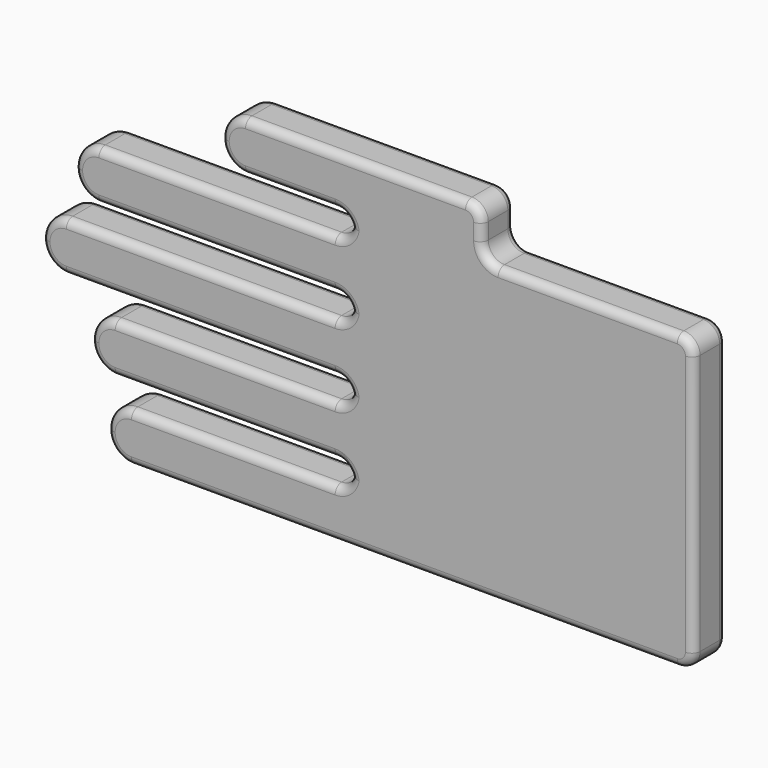
from build123d import *

# Parameters (mm, degrees)
F0_W          = 43.18
F0_H          = 7.62
F0_W_2        = 48.26
F0_W_3        = 40.64
F0_W_4        = 38.1
F1_DEPTH      = 6.35
F2_R          = 3.80999
F3_T1_DEPTH   = 6.35
F3_T3_DEPTH   = 19.05
F4_T3_DEPTH   = 13.97001
F4_T6_DEPTH   = 13.97001
F4_T9_DEPTH   = 36.83001
F4_T12_DEPTH  = 41.91001
F4_T15_DEPTH  = 34.29001
F4_T18_DEPTH  = 34.29001
F4_T21_DEPTH  = 41.91001
F4_T24_DEPTH  = 36.83001
F4_T27_DEPTH  = 34.29001
F4_T30_DEPTH  = 2e-05
F4_T33_DEPTH  = 2e-05
F4_T36_ANGLE  = 90
F4_T39_DEPTH  = 34.29001
F4_T42_ANGLE  = 89.9999999979
F4_T45_DEPTH  = 2.54
F4_T48_ANGLE  = 90.0000000056
F4_T51_DEPTH  = 27.94
F4_T54_ANGLE  = 89.9999999979
F4_T57_DEPTH  = 40.64
F4_T60_ANGLE  = 89.9999999979
F4_T63_DEPTH  = 85.09001
F4_T66_ANGLE  = 90
F4_T69_DEPTH  = 2e-05
F4_T72_ANGLE  = 90
F4_T75_DEPTH  = 31.75001
F4_T78_ANGLE  = 147.1624691834
F4_T82_ANGLE  = 147.1624691834
F4_S83_R      = 2.54
F4_T84_DEPTH  = 7
F4_T87_ANGLE  = 147.1624691834
F4_S88_R      = 2.54
F4_T89_DEPTH  = 7
F4_T92_ANGLE  = 147.1624691834
F4_T96_ANGLE  = 90
F4_T99_DEPTH  = 2e-05
F4_T102_ANGLE = 90
F4_T105_ANGLE = 147.1624691834
F4_S106_R     = 2.54
F4_T107_DEPTH = 7
F4_T110_ANGLE = 147.1624691834
F4_T114_ANGLE = 147.1624691834
F4_T118_ANGLE = 147.1624691834
F4_S119_R     = 2.54
F4_T120_DEPTH = 7
F4_T123_DEPTH = 41.91001
F4_T126_ANGLE = 90
F4_T129_DEPTH = 2e-05
F4_T132_ANGLE = 90
F4_T135_ANGLE = 147.1624691834
F4_S136_R     = 2.54
F4_T137_DEPTH = 7
F4_T140_ANGLE = 147.1624691834
F4_T144_ANGLE = 147.1624691834
F4_T148_ANGLE = 147.1624691834
F4_S149_R     = 2.54
F4_T150_DEPTH = 7
F4_T153_DEPTH = 36.83001
F4_T156_ANGLE = 90
F4_T159_DEPTH = 2e-05
F4_T162_ANGLE = 90
F4_T165_ANGLE = 147.1624691834
F4_S166_R     = 2.54
F4_T167_DEPTH = 6
F4_T170_ANGLE = 147.1624691834
F4_T174_ANGLE = 147.1624691834
F4_T178_ANGLE = 147.1624691834
F4_S179_R     = 2.54
F4_T180_DEPTH = 7
F4_T183_ANGLE = 90
F4_T186_ANGLE = 90
F4_T189_ANGLE = 90
F4_T192_DEPTH = 34.29001
F4_T195_ANGLE = 89.9999999979
F4_T198_DEPTH = 2.54
F4_T201_ANGLE = 90.0000000056
F4_T204_DEPTH = 27.94
F4_T207_ANGLE = 89.9999999979
F4_T210_DEPTH = 40.64
F4_T213_ANGLE = 89.9999999979
F4_T216_DEPTH = 85.09001
F4_T219_ANGLE = 90
F4_T222_DEPTH = 2e-05
F4_T225_ANGLE = 90
F4_T228_DEPTH = 31.75001
F4_T231_ANGLE = 147.1624691834
F4_T235_ANGLE = 147.1624691834
F4_S236_R     = 2.54
F4_T237_DEPTH = 7
F4_T240_ANGLE = 147.1624691834
F4_S241_R     = 2.54
F4_T242_DEPTH = 7
F4_T245_ANGLE = 147.1624691834
F4_T249_ANGLE = 90
F4_T252_DEPTH = 2e-05
F4_T255_ANGLE = 90
F4_T258_DEPTH = 34.29001
F4_T261_ANGLE = 147.1624691834
F4_S262_R     = 2.54
F4_T263_DEPTH = 7
F4_T266_ANGLE = 147.1624691834
F4_T270_ANGLE = 147.1624691834
F4_T274_ANGLE = 147.1624691834
F4_S275_R     = 2.54
F4_T276_DEPTH = 7
F4_T279_DEPTH = 41.91001
F4_T282_ANGLE = 90
F4_T285_DEPTH = 2e-05
F4_T288_ANGLE = 90
F4_T291_ANGLE = 147.1624691834
F4_S292_R     = 2.54
F4_T293_DEPTH = 7
F4_T296_ANGLE = 147.1624691834
F4_T300_ANGLE = 147.1624691834
F4_T304_ANGLE = 147.1624691834
F4_S305_R     = 2.54
F4_T306_DEPTH = 7
F4_T309_DEPTH = 36.83001
F4_T312_ANGLE = 90
F4_T315_DEPTH = 2e-05
F4_T318_ANGLE = 90
F4_T321_ANGLE = 147.1624691834
F4_S322_R     = 2.54
F4_T323_DEPTH = 6
F4_T326_ANGLE = 147.1624691834
F4_T330_ANGLE = 147.1624691834
F4_T334_ANGLE = 147.1624691834
F4_S335_R     = 2.54
F4_T336_DEPTH = 7
F4_T340_ANGLE = 147.1624691834
F4_S342_R     = 2.54
F4_T343_DEPTH = 7
F4_T346_ANGLE = 147.1624691834
F4_S347_R     = 2.54
F4_T348_DEPTH = 7
F4_T354_ANGLE = 147.1624691834
F4_S356_R     = 2.54
F4_T357_DEPTH = 7
F4_T360_ANGLE = 147.1624691834
F4_S361_R     = 2.54
F4_T362_DEPTH = 7
F4_T368_ANGLE = 147.1624691834
F4_S370_R     = 2.54
F4_T371_DEPTH = 7
F4_T374_ANGLE = 147.1624691834
F4_S375_R     = 2.54
F4_T376_DEPTH = 7
F4_T382_ANGLE = 147.1624691834
F4_S384_R     = 2.54
F4_T385_DEPTH = 6
F4_T388_ANGLE = 147.1624691834
F4_S389_R     = 2.54
F4_T390_DEPTH = 7
F4_T396_ANGLE = 147.1624691834
F4_S398_R     = 2.54
F4_T399_DEPTH = 7
F4_T402_ANGLE = 147.1624691834
F4_S403_R     = 2.54
F4_T404_DEPTH = 7
F4_T410_ANGLE = 147.1624691834
F4_S412_R     = 2.54
F4_T413_DEPTH = 7
F4_T416_ANGLE = 147.1624691834
F4_S417_R     = 2.54
F4_T418_DEPTH = 7
F4_T424_ANGLE = 147.1624691834
F4_S426_R     = 2.54
F4_T427_DEPTH = 7
F4_T430_ANGLE = 147.1624691834
F4_S431_R     = 2.54
F4_T432_DEPTH = 7
F4_T438_ANGLE = 147.1624691834
F4_S440_R     = 2.54
F4_T441_DEPTH = 6
F4_T444_ANGLE = 147.1624691834
F4_S445_R     = 2.54
F4_T446_DEPTH = 7


# Not quite as in the source:
# - a fillet or chamfer that OpenCascade refuses, or shapes differently, is made with other operations: its cross-section is extruded or revolved along the edge and cut away or added
# - a fillet or chamfer is up to 0.001 mm smaller than in the source, because OpenCascade refuses the exact size


with BuildPart() as f1:
    # F0 (on Front) → F1 (new body)
    with BuildSketch(Plane.XZ):
        Polygon((-50.9331456017, 28.2677418992), (-30.6131456017, 28.2677418992), (-10.2931456017, 28.2677418992), (-10.2931456017, 35.8877418992), (-50.9331456017, 35.8877418992), align=None)
        with Locations((-52.2031456017, 20.6477418992)):
            Rectangle(F0_W, F0_H)
        with Locations((-54.7431456017, 9.2177418992)):
            Rectangle(F0_W_2, F0_H)
        with Locations((-50.9331456017, -2.2122581008)):
            Rectangle(F0_W_3, F0_H)
        with Locations((-49.6631456017, -13.6422581008)):
            Rectangle(F0_W_4, F0_H)
        Polygon((-10.2931456017, 28.2677418992), (-30.6131456017, 28.2677418992), (-30.6131456017, 24.4577418992), (-30.6131456017, 16.8377418992), (-30.6131456017, 13.0277418992), (-30.6131456017, 5.4077418992), (-30.6131456017, 1.5977418992), (-30.6131456017, -6.0222581008), (-30.6131456017, -9.8322581008), (-30.6131456017, -17.4522581008), (22.7268543983, -17.4522581008), (22.7268543983, 28.2677418992), align=None)
    extrude(amount=F1_DEPTH)

    # F2 (radius 3.81 in the source; OpenCascade refuses exactly that, so slightly less here)
    f2_edges = [f1.edges().sort_by_distance(p)[0] for p in [
        (-73.793146, -3.175, 24.457742),
        (-73.793146, -3.175, 16.837742),
        (-78.873146, -3.175, 5.407742),
        (-78.873146, -3.175, 13.027742),
        (-71.253146, -3.175, -6.022258),
        (-71.253146, -3.175, 1.597742),
        (-68.713146, -3.175, -9.832258),
        (-68.713146, -3.175, -17.452258),
        (-50.933146, -3.175, 35.887742),
        (-50.933146, -3.175, 28.267742),
    ]]
    fillet(f2_edges, radius=F2_R)

    # F3: fillet of radius 2.54 on 12 edges, made by hand

    # F3_s2 → F3_t1 (join)
    with BuildSketch(Plane.XZ):
        with BuildLine():
            ThreePointArc((-10.2931456017, 30.8077418992), (-9.549196826, 29.011690675), (-7.7531456017, 28.2677418992))
            Line((-7.7531456017, 28.2677418992), (-10.2931456017, 28.2677418992))
            Line((-10.2931456017, 28.2677418992), (-10.2931456017, 30.8077418992))
        make_face()
        with BuildLine():
            ThreePointArc((-33.1531456017, 28.2677418992), (-31.3570943775, 27.5237931234), (-30.6131456017, 25.7277418992))
            Line((-30.6131456017, 25.7277418992), (-30.6131456017, 28.2677418992))
            Line((-30.6131456017, 28.2677418992), (-33.1531456017, 28.2677418992))
        make_face()
        with BuildLine():
            ThreePointArc((-33.1531456017, 16.8377418992), (-31.3570943775, 16.0937931234), (-30.6131456017, 14.2977418992))
            Line((-30.6131456017, 14.2977418992), (-30.6131456017, 16.8377418992))
            Line((-30.6131456017, 16.8377418992), (-33.1531456017, 16.8377418992))
        make_face()
        with BuildLine():
            ThreePointArc((-33.1531456017, 5.4077418992), (-31.3570943775, 4.6637931234), (-30.6131456017, 2.8677418992))
            Line((-30.6131456017, 2.8677418992), (-30.6131456017, 5.4077418992))
            Line((-30.6131456017, 5.4077418992), (-33.1531456017, 5.4077418992))
        make_face()
        with BuildLine():
            ThreePointArc((-30.6131456017, -8.5622581008), (-31.3570943775, -6.7662068766), (-33.1531456017, -6.0222581008))
            Line((-33.1531456017, -6.0222581008), (-30.6131456017, -6.0222581008))
            Line((-30.6131456017, -6.0222581008), (-30.6131456017, -8.5622581008))
        make_face()
        with BuildLine():
            ThreePointArc((-30.6131456017, 26.9977418992), (-31.3570943775, 25.201690675), (-33.1531456017, 24.4577418992))
            Line((-33.1531456017, 24.4577418992), (-30.6131456017, 24.4577418992))
            Line((-30.6131456017, 24.4577418992), (-30.6131456017, 26.9977418992))
        make_face()
        with BuildLine():
            ThreePointArc((-30.6131456017, 15.5677418992), (-31.3570943775, 13.771690675), (-33.1531456017, 13.0277418992))
            Line((-33.1531456017, 13.0277418992), (-30.6131456017, 13.0277418992))
            Line((-30.6131456017, 13.0277418992), (-30.6131456017, 15.5677418992))
        make_face()
        with BuildLine():
            ThreePointArc((-30.6131456017, 4.1377418992), (-31.3570943775, 2.341690675), (-33.1531456017, 1.5977418992))
            Line((-33.1531456017, 1.5977418992), (-30.6131456017, 1.5977418992))
            Line((-30.6131456017, 1.5977418992), (-30.6131456017, 4.1377418992))
        make_face()
        with BuildLine():
            ThreePointArc((-33.1531456017, -9.8322581008), (-31.3570943775, -9.088309325), (-30.6131456017, -7.2922581008))
            Line((-30.6131456017, -7.2922581008), (-30.6131456017, -9.8322581008))
            Line((-30.6131456017, -9.8322581008), (-33.1531456017, -9.8322581008))
        make_face()
    extrude(amount=F3_T1_DEPTH)

    # F3_s4 → F3_t3 (cut)
    with BuildSketch(Plane.XZ.offset(-6.35)):
        with BuildLine():
            ThreePointArc((-12.8331456017, 35.8877418992), (-11.0370943775, 35.1437931234), (-10.2931456017, 33.3477418992))
            Line((-10.2931456017, 33.3477418992), (-10.2931456017, 35.8877418992))
            Line((-10.2931456017, 35.8877418992), (-12.8331456017, 35.8877418992))
        make_face()
        with BuildLine():
            ThreePointArc((20.1868543983, 28.2677418992), (21.9829056225, 27.5237931234), (22.7268543983, 25.7277418992))
            Line((22.7268543983, 25.7277418992), (22.7268543983, 28.2677418992))
            Line((22.7268543983, 28.2677418992), (20.1868543983, 28.2677418992))
        make_face()
        with BuildLine():
            ThreePointArc((22.7268543983, -14.9122581008), (21.9829056225, -16.708309325), (20.1868543983, -17.4522581008))
            Line((20.1868543983, -17.4522581008), (22.7268543983, -17.4522581008))
            Line((22.7268543983, -17.4522581008), (22.7268543983, -14.9122581008))
        make_face()
    extrude(amount=F3_T3_DEPTH, mode=Mode.SUBTRACT)

    # F4: fillet of radius 1.27 on 80 edges, made by hand


with BuildPart() as f4_tool1:
    # F4_s2 → F4_t3 (new body)
    with BuildSketch(Plane.YZ.offset(-47.1231556017)):
        with BuildLine():
            ThreePointArc((-6.35, 29.5377418992), (-5.9780256121, 28.6397162871), (-5.08, 28.2677418992))
            Line((-5.08, 28.2677418992), (-6.35, 28.2677418992))
            Line((-6.35, 28.2677418992), (-6.35, 29.5377418992))
        make_face()
    extrude(amount=F4_T3_DEPTH)


with BuildPart() as f4_tool4:
    # F4_s5 → F4_t6 (new body)
    with BuildSketch(Plane.YZ.offset(-47.1231556017)):
        with BuildLine():
            ThreePointArc((0, 29.5377418992), (-0.3719743879, 28.6397162871), (-1.27, 28.2677418992))
            Line((-1.27, 28.2677418992), (0, 28.2677418992))
            Line((0, 28.2677418992), (0, 29.5377418992))
        make_face()
    extrude(amount=F4_T6_DEPTH)


with BuildPart() as f4_tool7:
    # F4_s8 → F4_t9 (new body)
    with BuildSketch(Plane.YZ.offset(-33.1531456017)):
        with BuildLine():
            ThreePointArc((-6.35, 23.1877418992), (-5.9780256121, 24.0857675113), (-5.08, 24.4577418992))
            Line((-5.08, 24.4577418992), (-6.35, 24.4577418992))
            Line((-6.35, 24.4577418992), (-6.35, 23.1877418992))
        make_face()
    extrude(amount=-F4_T9_DEPTH)


with BuildPart() as f4_tool10:
    # F4_s11 → F4_t12 (new body)
    with BuildSketch(Plane.YZ.offset(-33.1531456017)):
        with BuildLine():
            ThreePointArc((-6.35, 11.7577418992), (-5.9780256121, 12.6557675113), (-5.08, 13.0277418992))
            Line((-5.08, 13.0277418992), (-6.35, 13.0277418992))
            Line((-6.35, 13.0277418992), (-6.35, 11.7577418992))
        make_face()
    extrude(amount=-F4_T12_DEPTH)


with BuildPart() as f4_tool13:
    # F4_s14 → F4_t15 (new body)
    with BuildSketch(Plane.YZ.offset(-67.4431556017)):
        with BuildLine():
            ThreePointArc((0, -4.7522581008), (-0.3719743879, -5.6502837129), (-1.27, -6.0222581008))
            Line((-1.27, -6.0222581008), (0, -6.0222581008))
            Line((0, -6.0222581008), (0, -4.7522581008))
        make_face()
    extrude(amount=F4_T15_DEPTH)


with BuildPart() as f4_tool16:
    # F4_s17 → F4_t18 (new body)
    with BuildSketch(Plane.YZ.offset(-33.1531456017)):
        with BuildLine():
            ThreePointArc((0, 0.3277418992), (-0.3719743879, 1.2257675113), (-1.27, 1.5977418992))
            Line((-1.27, 1.5977418992), (0, 1.5977418992))
            Line((0, 1.5977418992), (0, 0.3277418992))
        make_face()
    extrude(amount=-F4_T18_DEPTH)


with BuildPart() as f4_tool19:
    # F4_s20 → F4_t21 (new body)
    with BuildSketch(Plane.YZ.offset(-33.1531456017)):
        with BuildLine():
            ThreePointArc((0, 11.7577418992), (-0.3719743879, 12.6557675113), (-1.27, 13.0277418992))
            Line((-1.27, 13.0277418992), (0, 13.0277418992))
            Line((0, 13.0277418992), (0, 11.7577418992))
        make_face()
    extrude(amount=-F4_T21_DEPTH)


with BuildPart() as f4_tool22:
    # F4_s23 → F4_t24 (new body)
    with BuildSketch(Plane.YZ.offset(-33.1531456017)):
        with BuildLine():
            ThreePointArc((0, 23.1877418992), (-0.3719743879, 24.0857675113), (-1.27, 24.4577418992))
            Line((-1.27, 24.4577418992), (0, 24.4577418992))
            Line((0, 24.4577418992), (0, 23.1877418992))
        make_face()
    extrude(amount=-F4_T24_DEPTH)


with BuildPart() as f4_tool25:
    # F4_s26 → F4_t27 (new body)
    with BuildSketch(Plane.YZ.offset(-67.4431556017)):
        with BuildLine():
            ThreePointArc((-6.35, -4.7522581008), (-5.9780256121, -5.6502837129), (-5.08, -6.0222581008))
            Line((-5.08, -6.0222581008), (-6.35, -6.0222581008))
            Line((-6.35, -6.0222581008), (-6.35, -4.7522581008))
        make_face()
    extrude(amount=F4_T27_DEPTH)


with BuildPart() as f4_tool28:
    # F4_s29 → F4_t30 (new body)
    with BuildSketch(Plane.XY.offset(32.0777518992)):
        with BuildLine():
            ThreePointArc((-50.9331456017, -1.27), (-50.5611712139, -0.3719743879), (-49.6631456017, 0))
            Line((-49.6631456017, 0), (-50.9331456017, 0))
            Line((-50.9331456017, 0), (-50.9331456017, -1.27))
        make_face()
    extrude(amount=-F4_T30_DEPTH)


with BuildPart() as f4_tool31:
    # F4_s32 → F4_t33 (new body)
    with BuildSketch(Plane.XY.offset(32.0777518992)):
        with BuildLine():
            ThreePointArc((-50.9331456017, -5.08), (-50.5611712139, -5.9780256121), (-49.6631456017, -6.35))
            Line((-49.6631456017, -6.35), (-50.9331456017, -6.35))
            Line((-50.9331456017, -6.35), (-50.9331456017, -5.08))
        make_face()
    extrude(amount=-F4_T33_DEPTH)


with BuildPart() as f4_tool34:
    # F4_s35 → F4_t36 (revolve)
    with BuildSketch(Plane.XY.offset(32.0777518992)):
        with BuildLine():
            ThreePointArc((-49.6631456017, 0), (-50.5611712139, -0.3719743879), (-50.9331456017, -1.27))
            Line((-50.9331456017, -1.27), (-50.9331456017, 0))
            Line((-50.9331456017, 0), (-49.6631456017, 0))
        make_face()
    revolve(axis=Axis((-47.1231556017, 0, 32.0777518992), (0, 1, 0)), revolution_arc=F4_T36_ANGLE)


with BuildPart() as f4_tool37:
    # F4_s38 → F4_t39 (new body)
    with BuildSketch(Plane.YZ.offset(-12.8331456017)):
        with BuildLine():
            ThreePointArc((0, 34.6177418992), (-0.3719743879, 35.5157675113), (-1.27, 35.8877418992))
            Line((-1.27, 35.8877418992), (0, 35.8877418992))
            Line((0, 35.8877418992), (0, 34.6177418992))
        make_face()
    extrude(amount=-F4_T39_DEPTH)


with BuildPart() as f4_tool40:
    # F4_s41 → F4_t42 (revolve)
    with BuildSketch(Plane.YZ.offset(-12.8331456017)):
        with BuildLine():
            ThreePointArc((0, 34.6177418992), (-0.3719743879, 35.5157675113), (-1.27, 35.8877418992))
            Line((-1.27, 35.8877418992), (0, 35.8877418992))
            Line((0, 35.8877418992), (0, 34.6177418992))
        make_face()
    revolve(axis=Axis((-12.8331456017, 0, 33.3477418992), (0, 1, 0)), revolution_arc=F4_T42_ANGLE)


with BuildPart() as f4_tool43:
    # F4_s44 → F4_t45 (new body)
    with BuildSketch(Plane.XY.offset(30.8077418992)):
        with BuildLine():
            ThreePointArc((-11.5631456017, 0), (-10.6651199896, -0.3719743879), (-10.2931456017, -1.27))
            Line((-10.2931456017, -1.27), (-10.2931456017, 0))
            Line((-10.2931456017, 0), (-11.5631456017, 0))
        make_face()
    extrude(amount=F4_T45_DEPTH)


with BuildPart() as f4_tool46:
    # F4_s47 → F4_t48 (revolve)
    with BuildSketch(Plane.XY.offset(30.8077418991)):
        with BuildLine():
            ThreePointArc((-11.5631456017, 0), (-10.6651199896, -0.3719743879), (-10.2931456017, -1.27))
            Line((-10.2931456017, -1.27), (-10.2931456017, 0))
            Line((-10.2931456017, 0), (-11.5631456017, 0))
        make_face()
    revolve(axis=Axis((-7.7531456018, 0, 30.8077418991), (0, -1, 0)), revolution_arc=F4_T48_ANGLE)


with BuildPart() as f4_tool49:
    # F4_s50 → F4_t51 (new body)
    with BuildSketch(Plane.YZ.offset(20.1868543983)):
        with BuildLine():
            ThreePointArc((0, 26.9977418992), (-0.3719743879, 27.8957675113), (-1.27, 28.2677418992))
            Line((-1.27, 28.2677418992), (0, 28.2677418992))
            Line((0, 28.2677418992), (0, 26.9977418992))
        make_face()
    extrude(amount=-F4_T51_DEPTH)


with BuildPart() as f4_tool52:
    # F4_s53 → F4_t54 (revolve)
    with BuildSketch(Plane.YZ.offset(20.1868543983)):
        with BuildLine():
            ThreePointArc((0, 26.9977418992), (-0.3719743879, 27.8957675113), (-1.27, 28.2677418992))
            Line((-1.27, 28.2677418992), (0, 28.2677418992))
            Line((0, 28.2677418992), (0, 26.9977418992))
        make_face()
    revolve(axis=Axis((20.1868543983, 0, 25.7277418992), (0, 1, 0)), revolution_arc=F4_T54_ANGLE)


with BuildPart() as f4_tool55:
    # F4_s56 → F4_t57 (new body)
    with BuildSketch(Plane.XY.offset(-14.9122581008)):
        with BuildLine():
            ThreePointArc((21.4568543983, 0), (22.3548800104, -0.3719743879), (22.7268543983, -1.27))
            Line((22.7268543983, -1.27), (22.7268543983, 0))
            Line((22.7268543983, 0), (21.4568543983, 0))
        make_face()
    extrude(amount=F4_T57_DEPTH)


with BuildPart() as f4_tool58:
    # F4_s59 → F4_t60 (revolve)
    with BuildSketch(Plane.XY.offset(-14.9122581008)):
        with BuildLine():
            ThreePointArc((21.4568543983, 0), (22.3548800104, -0.3719743879), (22.7268543983, -1.27))
            Line((22.7268543983, -1.27), (22.7268543983, 0))
            Line((22.7268543983, 0), (21.4568543983, 0))
        make_face()
    revolve(axis=Axis((20.1868543983, 0, -14.9122581008), (0, 1, 0)), revolution_arc=F4_T60_ANGLE)


with BuildPart() as f4_tool61:
    # F4_s62 → F4_t63 (new body)
    with BuildSketch(Plane.YZ.offset(-64.9031556017)):
        with BuildLine():
            ThreePointArc((0, -16.1822581008), (-0.3719743879, -17.0802837129), (-1.27, -17.4522581008))
            Line((-1.27, -17.4522581008), (0, -17.4522581008))
            Line((0, -17.4522581008), (0, -16.1822581008))
        make_face()
    extrude(amount=F4_T63_DEPTH)


with BuildPart() as f4_tool64:
    # F4_s65 → F4_t66 (revolve)
    with BuildSketch(Plane.XY.offset(-13.6422681008)):
        with BuildLine():
            ThreePointArc((-67.4431456017, 0), (-68.3411712139, -0.3719743879), (-68.7131456017, -1.27))
            Line((-68.7131456017, -1.27), (-68.7131456017, 0))
            Line((-68.7131456017, 0), (-67.4431456017, 0))
        make_face()
    revolve(axis=Axis((-64.9031556017, 0, -13.6422681008), (0, -1, 0)), revolution_arc=F4_T66_ANGLE)


with BuildPart() as f4_tool67:
    # F4_s68 → F4_t69 (new body)
    with BuildSketch(Plane.XY.offset(-13.6422481008)):
        with BuildLine():
            ThreePointArc((-67.4431456017, 0), (-68.3411712139, -0.3719743879), (-68.7131456017, -1.27))
            Line((-68.7131456017, -1.27), (-68.7131456017, 0))
            Line((-68.7131456017, 0), (-67.4431456017, 0))
        make_face()
    extrude(amount=-F4_T69_DEPTH)


with BuildPart() as f4_tool70:
    # F4_s71 → F4_t72 (revolve)
    with BuildSketch(Plane.YZ.offset(-64.9031556017)):
        with BuildLine():
            ThreePointArc((0, -11.1022581008), (-0.3719743879, -10.2042324887), (-1.27, -9.8322581008))
            Line((-1.27, -9.8322581008), (0, -9.8322581008))
            Line((0, -9.8322581008), (0, -11.1022581008))
        make_face()
    revolve(axis=Axis((-64.9031556017, 0, -13.6422481008), (0, -1, 0)), revolution_arc=F4_T72_ANGLE)


with BuildPart() as f4_tool73:
    # F4_s74 → F4_t75 (new body)
    with BuildSketch(Plane.YZ.offset(-33.1531456017)):
        with BuildLine():
            ThreePointArc((0, -11.1022581008), (-0.3719743879, -10.2042324887), (-1.27, -9.8322581008))
            Line((-1.27, -9.8322581008), (0, -9.8322581008))
            Line((0, -9.8322581008), (0, -11.1022581008))
        make_face()
    extrude(amount=-F4_T75_DEPTH)


with BuildPart() as f4_tool76:
    # F4_s77 → F4_t78 (revolve)
    with BuildSketch(Plane.YZ.offset(-33.1531456017)):
        with BuildLine():
            ThreePointArc((0, -11.1022581008), (-0.3719743879, -10.2042324887), (-1.27, -9.8322581008))
            Line((-1.27, -9.8322581008), (0, -9.8322581008))
            Line((0, -9.8322581008), (0, -11.1022581008))
        make_face()
    revolve(axis=Axis((-33.1531456017, 0, -7.2922581008), (0, -1, 0)), revolution_arc=F4_T78_ANGLE)

    split(bisect_by=Plane.XY.offset(-9.8322581008), keep=Keep.BOTTOM)


with BuildPart() as f4_tool80:
    # F4_s81 → F4_t82 (revolve)
    with BuildSketch(Plane.YZ.offset(-33.1531456017)):
        with BuildLine():
            ThreePointArc((0, -11.1022581008), (-0.3719743879, -10.2042324887), (-1.27, -9.8322581008))
            Line((-1.27, -9.8322581008), (0, -9.8322581008))
            Line((0, -9.8322581008), (0, -11.1022581008))
        make_face()
    revolve(axis=Axis((-33.1531456017, 0, -7.2922581008), (0, -1, 0)), revolution_arc=F4_T82_ANGLE)

    # F4_s83 → F4_t84 (intersect, symmetric)
    with BuildSketch(Plane.XZ.offset(1.1)):
        with Locations((-33.1531456017, -8.5622581008)):
            Circle(F4_S83_R)
    extrude(amount=F4_T84_DEPTH, both=True, mode=Mode.INTERSECT)


with BuildPart() as f4_tool85:
    # F4_s86 → F4_t87 (revolve)
    with BuildSketch(Plane(origin=(-27.305713574, 0, -17.6226570753), x_dir=(0, 1, 0), z_dir=(-0.8402115846, 0, -0.5422586957))):
        with BuildLine():
            ThreePointArc((0, -6.9734730442), (-0.3719743879, -7.8714986563), (-1.27, -8.2434730442))
            Line((-1.27, -8.2434730442), (0, -8.2434730442))
            Line((0, -8.2434730442), (0, -6.9734730442))
        make_face()
    revolve(axis=Axis((-33.1531456017, 0, -8.5622581008), (0, -1, 0)), revolution_arc=F4_T87_ANGLE)

    # F4_s88 → F4_t89 (intersect, symmetric)
    with BuildSketch(Plane.XZ.offset(1.1)):
        with Locations((-33.1531456017, -7.2922581008)):
            Circle(F4_S88_R)
    extrude(amount=F4_T89_DEPTH, both=True, mode=Mode.INTERSECT)


with BuildPart() as f4_tool90:
    # F4_s91 → F4_t92 (revolve)
    with BuildSketch(Plane(origin=(-27.305713574, 0, -17.6226570753), x_dir=(0, 1, 0), z_dir=(-0.8402115846, 0, -0.5422586957))):
        with BuildLine():
            ThreePointArc((0, -6.9734730442), (-0.3719743879, -7.8714986563), (-1.27, -8.2434730442))
            Line((-1.27, -8.2434730442), (0, -8.2434730442))
            Line((0, -8.2434730442), (0, -6.9734730442))
        make_face()
    revolve(axis=Axis((-33.1531456017, 0, -8.5622581008), (0, -1, 0)), revolution_arc=F4_T92_ANGLE)

    split(bisect_by=Plane.XY.offset(-6.0222581008), keep=Keep.TOP)


with BuildPart() as f4_tool94:
    # F4_s95 → F4_t96 (revolve)
    with BuildSketch(Plane.XY.offset(-2.2122681008)):
        with BuildLine():
            ThreePointArc((-69.9831456017, 0), (-70.8811712139, -0.3719743879), (-71.2531456017, -1.27))
            Line((-71.2531456017, -1.27), (-71.2531456017, 0))
            Line((-71.2531456017, 0), (-69.9831456017, 0))
        make_face()
    revolve(axis=Axis((-67.4431556017, 0, -2.2122681008), (0, -1, 0)), revolution_arc=F4_T96_ANGLE)


with BuildPart() as f4_tool97:
    # F4_s98 → F4_t99 (new body)
    with BuildSketch(Plane.XY.offset(-2.2122481008)):
        with BuildLine():
            ThreePointArc((-69.9831456017, 0), (-70.8811712139, -0.3719743879), (-71.2531456017, -1.27))
            Line((-71.2531456017, -1.27), (-71.2531456017, 0))
            Line((-71.2531456017, 0), (-69.9831456017, 0))
        make_face()
    extrude(amount=-F4_T99_DEPTH)


with BuildPart() as f4_tool100:
    # F4_s101 → F4_t102 (revolve)
    with BuildSketch(Plane.YZ.offset(-67.4431556017)):
        with BuildLine():
            ThreePointArc((0, 0.3277418992), (-0.3719743879, 1.2257675113), (-1.27, 1.5977418992))
            Line((-1.27, 1.5977418992), (0, 1.5977418992))
            Line((0, 1.5977418992), (0, 0.3277418992))
        make_face()
    revolve(axis=Axis((-67.4431556017, 0, -2.2122481008), (0, -1, 0)), revolution_arc=F4_T102_ANGLE)


with BuildPart() as f4_tool103:
    # F4_s104 → F4_t105 (revolve)
    with BuildSketch(Plane(origin=(-25.2898507304, 0, 16.3216524519), x_dir=(0, 1, 0), z_dir=(-0.8402115846, 0, 0.5422586957))):
        with BuildLine():
            ThreePointArc((0, 10.6910028132), (-0.3719743879, 11.5890284253), (-1.27, 11.9610028132))
            Line((-1.27, 11.9610028132), (0, 11.9610028132))
            Line((0, 11.9610028132), (0, 10.6910028132))
        make_face()
    revolve(axis=Axis((-33.1531456017, 0, 4.1377418992), (0, 1, 0)), revolution_arc=F4_T105_ANGLE)

    # F4_s106 → F4_t107 (intersect, symmetric)
    with BuildSketch(Plane.XZ.offset(1.1)):
        with Locations((-33.1531456017, 2.8677418992)):
            Circle(F4_S106_R)
    extrude(amount=F4_T107_DEPTH, both=True, mode=Mode.INTERSECT)


with BuildPart() as f4_tool108:
    # F4_s109 → F4_t110 (revolve)
    with BuildSketch(Plane(origin=(-25.2898507304, 0, 16.3216524519), x_dir=(0, 1, 0), z_dir=(-0.8402115846, 0, 0.5422586957))):
        with BuildLine():
            ThreePointArc((0, 10.6910028132), (-0.3719743879, 11.5890284253), (-1.27, 11.9610028132))
            Line((-1.27, 11.9610028132), (0, 11.9610028132))
            Line((0, 11.9610028132), (0, 10.6910028132))
        make_face()
    revolve(axis=Axis((-33.1531456017, 0, 4.1377418992), (0, 1, 0)), revolution_arc=F4_T110_ANGLE)

    split(bisect_by=Plane.XY.offset(1.5977418992), keep=Keep.BOTTOM)


with BuildPart() as f4_tool112:
    # F4_s113 → F4_t114 (revolve)
    with BuildSketch(Plane.YZ.offset(-33.1531456017)):
        with BuildLine():
            ThreePointArc((0, 6.6777418992), (-0.3719743879, 5.7797162871), (-1.27, 5.4077418992))
            Line((-1.27, 5.4077418992), (0, 5.4077418992))
            Line((0, 5.4077418992), (0, 6.6777418992))
        make_face()
    revolve(axis=Axis((-33.1531456017, 0, 2.8677418992), (0, 1, 0)), revolution_arc=F4_T114_ANGLE)

    split(bisect_by=Plane.XY.offset(5.4077418992), keep=Keep.TOP)


with BuildPart() as f4_tool116:
    # F4_s117 → F4_t118 (revolve)
    with BuildSketch(Plane.YZ.offset(-33.1531456017)):
        with BuildLine():
            ThreePointArc((0, 6.6777418992), (-0.3719743879, 5.7797162871), (-1.27, 5.4077418992))
            Line((-1.27, 5.4077418992), (0, 5.4077418992))
            Line((0, 5.4077418992), (0, 6.6777418992))
        make_face()
    revolve(axis=Axis((-33.1531456017, 0, 2.8677418992), (0, 1, 0)), revolution_arc=F4_T118_ANGLE)

    # F4_s119 → F4_t120 (intersect, symmetric)
    with BuildSketch(Plane.XZ.offset(1.1)):
        with Locations((-33.1531456017, 4.1377418992)):
            Circle(F4_S119_R)
    extrude(amount=F4_T120_DEPTH, both=True, mode=Mode.INTERSECT)


with BuildPart() as f4_tool121:
    # F4_s122 → F4_t123 (new body)
    with BuildSketch(Plane.YZ.offset(-75.0631556017)):
        with BuildLine():
            ThreePointArc((0, 6.6777418992), (-0.3719743879, 5.7797162871), (-1.27, 5.4077418992))
            Line((-1.27, 5.4077418992), (0, 5.4077418992))
            Line((0, 5.4077418992), (0, 6.6777418992))
        make_face()
    extrude(amount=F4_T123_DEPTH)


with BuildPart() as f4_tool124:
    # F4_s125 → F4_t126 (revolve)
    with BuildSketch(Plane.XY.offset(9.2177318992)):
        with BuildLine():
            ThreePointArc((-77.6031456017, 0), (-78.5011712139, -0.3719743879), (-78.8731456017, -1.27))
            Line((-78.8731456017, -1.27), (-78.8731456017, 0))
            Line((-78.8731456017, 0), (-77.6031456017, 0))
        make_face()
    revolve(axis=Axis((-75.0631556017, 0, 9.2177318992), (0, -1, 0)), revolution_arc=F4_T126_ANGLE)


with BuildPart() as f4_tool127:
    # F4_s128 → F4_t129 (new body)
    with BuildSketch(Plane.XY.offset(9.2177518992)):
        with BuildLine():
            ThreePointArc((-77.6031456017, 0), (-78.5011712139, -0.3719743879), (-78.8731456017, -1.27))
            Line((-78.8731456017, -1.27), (-78.8731456017, 0))
            Line((-78.8731456017, 0), (-77.6031456017, 0))
        make_face()
    extrude(amount=-F4_T129_DEPTH)


with BuildPart() as f4_tool130:
    # F4_s131 → F4_t132 (revolve)
    with BuildSketch(Plane.YZ.offset(-75.0631556017)):
        with BuildLine():
            ThreePointArc((0, 11.7577418992), (-0.3719743879, 12.6557675113), (-1.27, 13.0277418992))
            Line((-1.27, 13.0277418992), (0, 13.0277418992))
            Line((0, 13.0277418992), (0, 11.7577418992))
        make_face()
    revolve(axis=Axis((-75.0631556017, 0, 9.2177518992), (0, -1, 0)), revolution_arc=F4_T132_ANGLE)


with BuildPart() as f4_tool133:
    # F4_s134 → F4_t135 (revolve)
    with BuildSketch(Plane(origin=(-30.4974963244, 0, 19.6825810072), x_dir=(0, 1, 0), z_dir=(-0.8402115846, 0, 0.5422586957))):
        with BuildLine():
            ThreePointArc((0, 1.0873844007), (-0.3719743879, 1.9854100128), (-1.27, 2.3573844007))
            Line((-1.27, 2.3573844007), (0, 2.3573844007))
            Line((0, 2.3573844007), (0, 1.0873844007))
        make_face()
    revolve(axis=Axis((-33.1531456017, 0, 15.5677418992), (0, 1, 0)), revolution_arc=F4_T135_ANGLE)

    # F4_s136 → F4_t137 (intersect, symmetric)
    with BuildSketch(Plane.XZ.offset(1.1)):
        with Locations((-33.1531456017, 14.2977418992)):
            Circle(F4_S136_R)
    extrude(amount=F4_T137_DEPTH, both=True, mode=Mode.INTERSECT)


with BuildPart() as f4_tool138:
    # F4_s139 → F4_t140 (revolve)
    with BuildSketch(Plane(origin=(-30.4974963244, 0, 19.6825810072), x_dir=(0, 1, 0), z_dir=(-0.8402115846, 0, 0.5422586957))):
        with BuildLine():
            ThreePointArc((0, 1.0873844007), (-0.3719743879, 1.9854100128), (-1.27, 2.3573844007))
            Line((-1.27, 2.3573844007), (0, 2.3573844007))
            Line((0, 2.3573844007), (0, 1.0873844007))
        make_face()
    revolve(axis=Axis((-33.1531456017, 0, 15.5677418992), (0, 1, 0)), revolution_arc=F4_T140_ANGLE)

    split(bisect_by=Plane.XY.offset(13.0277418992), keep=Keep.BOTTOM)


with BuildPart() as f4_tool142:
    # F4_s143 → F4_t144 (revolve)
    with BuildSketch(Plane.YZ.offset(-33.1531456017)):
        with BuildLine():
            ThreePointArc((0, 18.1077418992), (-0.3719743879, 17.2097162871), (-1.27, 16.8377418992))
            Line((-1.27, 16.8377418992), (0, 16.8377418992))
            Line((0, 16.8377418992), (0, 18.1077418992))
        make_face()
    revolve(axis=Axis((-33.1531456017, 0, 14.2977418992), (0, 1, 0)), revolution_arc=F4_T144_ANGLE)

    split(bisect_by=Plane.XY.offset(16.8377418992), keep=Keep.TOP)


with BuildPart() as f4_tool146:
    # F4_s147 → F4_t148 (revolve)
    with BuildSketch(Plane.YZ.offset(-33.1531456017)):
        with BuildLine():
            ThreePointArc((0, 18.1077418992), (-0.3719743879, 17.2097162871), (-1.27, 16.8377418992))
            Line((-1.27, 16.8377418992), (0, 16.8377418992))
            Line((0, 16.8377418992), (0, 18.1077418992))
        make_face()
    revolve(axis=Axis((-33.1531456017, 0, 14.2977418992), (0, 1, 0)), revolution_arc=F4_T148_ANGLE)

    # F4_s149 → F4_t150 (intersect, symmetric)
    with BuildSketch(Plane.XZ.offset(1.1)):
        with Locations((-33.1531456017, 15.5677418992)):
            Circle(F4_S149_R)
    extrude(amount=F4_T150_DEPTH, both=True, mode=Mode.INTERSECT)


with BuildPart() as f4_tool151:
    # F4_s152 → F4_t153 (new body)
    with BuildSketch(Plane.YZ.offset(-69.9831556017)):
        with BuildLine():
            ThreePointArc((0, 18.1077418992), (-0.3719743879, 17.2097162871), (-1.27, 16.8377418992))
            Line((-1.27, 16.8377418992), (0, 16.8377418992))
            Line((0, 16.8377418992), (0, 18.1077418992))
        make_face()
    extrude(amount=F4_T153_DEPTH)


with BuildPart() as f4_tool154:
    # F4_s155 → F4_t156 (revolve)
    with BuildSketch(Plane.XY.offset(20.6477318992)):
        with BuildLine():
            ThreePointArc((-72.5231456017, 0), (-73.4211712139, -0.3719743879), (-73.7931456017, -1.27))
            Line((-73.7931456017, -1.27), (-73.7931456017, 0))
            Line((-73.7931456017, 0), (-72.5231456017, 0))
        make_face()
    revolve(axis=Axis((-69.9831556017, 0, 20.6477318992), (0, -1, 0)), revolution_arc=F4_T156_ANGLE)


with BuildPart() as f4_tool157:
    # F4_s158 → F4_t159 (new body)
    with BuildSketch(Plane.XY.offset(20.6477518992)):
        with BuildLine():
            ThreePointArc((-72.5231456017, 0), (-73.4211712139, -0.3719743879), (-73.7931456017, -1.27))
            Line((-73.7931456017, -1.27), (-73.7931456017, 0))
            Line((-73.7931456017, 0), (-72.5231456017, 0))
        make_face()
    extrude(amount=-F4_T159_DEPTH)


with BuildPart() as f4_tool160:
    # F4_s161 → F4_t162 (revolve)
    with BuildSketch(Plane.YZ.offset(-69.9831556017)):
        with BuildLine():
            ThreePointArc((0, 23.1877418992), (-0.3719743879, 24.0857675113), (-1.27, 24.4577418992))
            Line((-1.27, 24.4577418992), (0, 24.4577418992))
            Line((0, 24.4577418992), (0, 23.1877418992))
        make_face()
    revolve(axis=Axis((-69.9831556017, 0, 20.6477518992), (0, -1, 0)), revolution_arc=F4_T162_ANGLE)


with BuildPart() as f4_tool163:
    # F4_s164 → F4_t165 (revolve)
    with BuildSketch(Plane(origin=(-35.7051419185, 0, 23.0435095625), x_dir=(0, 1, 0), z_dir=(-0.8402115846, 0, 0.5422586957))):
        with BuildLine():
            ThreePointArc((0, -8.5162340118), (-0.3719743879, -7.6182083997), (-1.27, -7.2462340118))
            Line((-1.27, -7.2462340118), (0, -7.2462340118))
            Line((0, -7.2462340118), (0, -8.5162340118))
        make_face()
    revolve(axis=Axis((-33.1531456017, 0, 26.9977418992), (0, 1, 0)), revolution_arc=F4_T165_ANGLE)

    # F4_s166 → F4_t167 (intersect, symmetric)
    with BuildSketch(Plane.XZ.offset(1.1)):
        with Locations((-33.1531456017, 25.7277418992)):
            Circle(F4_S166_R)
    extrude(amount=F4_T167_DEPTH, both=True, mode=Mode.INTERSECT)


with BuildPart() as f4_tool168:
    # F4_s169 → F4_t170 (revolve)
    with BuildSketch(Plane(origin=(-35.7051419185, 0, 23.0435095625), x_dir=(0, 1, 0), z_dir=(-0.8402115846, 0, 0.5422586957))):
        with BuildLine():
            ThreePointArc((0, -8.5162340118), (-0.3719743879, -7.6182083997), (-1.27, -7.2462340118))
            Line((-1.27, -7.2462340118), (0, -7.2462340118))
            Line((0, -7.2462340118), (0, -8.5162340118))
        make_face()
    revolve(axis=Axis((-33.1531456017, 0, 26.9977418992), (0, 1, 0)), revolution_arc=F4_T170_ANGLE)

    split(bisect_by=Plane.XY.offset(24.4577418992), keep=Keep.BOTTOM)


with BuildPart() as f4_tool172:
    # F4_s173 → F4_t174 (revolve)
    with BuildSketch(Plane.YZ.offset(-33.1531456017)):
        with BuildLine():
            ThreePointArc((0, 29.5377418992), (-0.3719743879, 28.6397162871), (-1.27, 28.2677418992))
            Line((-1.27, 28.2677418992), (0, 28.2677418992))
            Line((0, 28.2677418992), (0, 29.5377418992))
        make_face()
    revolve(axis=Axis((-33.1531456017, 0, 25.7277418992), (0, 1, 0)), revolution_arc=F4_T174_ANGLE)

    split(bisect_by=Plane.XY.offset(28.2677418992), keep=Keep.TOP)


with BuildPart() as f4_tool176:
    # F4_s177 → F4_t178 (revolve)
    with BuildSketch(Plane.YZ.offset(-33.1531456017)):
        with BuildLine():
            ThreePointArc((0, 29.5377418992), (-0.3719743879, 28.6397162871), (-1.27, 28.2677418992))
            Line((-1.27, 28.2677418992), (0, 28.2677418992))
            Line((0, 28.2677418992), (0, 29.5377418992))
        make_face()
    revolve(axis=Axis((-33.1531456017, 0, 25.7277418992), (0, 1, 0)), revolution_arc=F4_T178_ANGLE)

    # F4_s179 → F4_t180 (intersect, symmetric)
    with BuildSketch(Plane.XZ.offset(1.1)):
        with Locations((-33.1531456017, 26.9977418992)):
            Circle(F4_S179_R)
    extrude(amount=F4_T180_DEPTH, both=True, mode=Mode.INTERSECT)


with BuildPart() as f4_tool181:
    # F4_s182 → F4_t183 (revolve)
    with BuildSketch(Plane.XY.offset(32.0777318992)):
        with BuildLine():
            ThreePointArc((-49.6631456017, 0), (-50.5611712139, -0.3719743879), (-50.9331456017, -1.27))
            Line((-50.9331456017, -1.27), (-50.9331456017, 0))
            Line((-50.9331456017, 0), (-49.6631456017, 0))
        make_face()
    revolve(axis=Axis((-47.1231556017, 0, 32.0777318992), (0, -1, 0)), revolution_arc=F4_T183_ANGLE)


with BuildPart() as f4_tool184:
    # F4_s185 → F4_t186 (revolve)
    with BuildSketch(Plane.XY.offset(32.0777518992)):
        with BuildLine():
            ThreePointArc((-50.9331456017, -5.08), (-50.5611712139, -5.9780256121), (-49.6631456017, -6.35))
            Line((-49.6631456017, -6.35), (-50.9331456017, -6.35))
            Line((-50.9331456017, -6.35), (-50.9331456017, -5.08))
        make_face()
    revolve(axis=Axis((-47.1231556017, -6.35, 32.0777518992), (0, 1, 0)), revolution_arc=F4_T186_ANGLE)


with BuildPart() as f4_tool187:
    # F4_s188 → F4_t189 (revolve)
    with BuildSketch(Plane.XY.offset(32.0777318992)):
        with BuildLine():
            ThreePointArc((-50.9331456017, -5.08), (-50.5611712139, -5.9780256121), (-49.6631456017, -6.35))
            Line((-49.6631456017, -6.35), (-50.9331456017, -6.35))
            Line((-50.9331456017, -6.35), (-50.9331456017, -5.08))
        make_face()
    revolve(axis=Axis((-47.1231556017, -6.35, 32.0777318992), (0, -1, 0)), revolution_arc=F4_T189_ANGLE)


with BuildPart() as f4_tool190:
    # F4_s191 → F4_t192 (new body)
    with BuildSketch(Plane.YZ.offset(-12.8331456017)):
        with BuildLine():
            ThreePointArc((-6.35, 34.6177418992), (-5.9780256121, 35.5157675113), (-5.08, 35.8877418992))
            Line((-5.08, 35.8877418992), (-6.35, 35.8877418992))
            Line((-6.35, 35.8877418992), (-6.35, 34.6177418992))
        make_face()
    extrude(amount=-F4_T192_DEPTH)


with BuildPart() as f4_tool193:
    # F4_s194 → F4_t195 (revolve)
    with BuildSketch(Plane.YZ.offset(-12.8331456017)):
        with BuildLine():
            ThreePointArc((-6.35, 34.6177418992), (-5.9780256121, 35.5157675113), (-5.08, 35.8877418992))
            Line((-5.08, 35.8877418992), (-6.35, 35.8877418992))
            Line((-6.35, 35.8877418992), (-6.35, 34.6177418992))
        make_face()
    revolve(axis=Axis((-12.8331456017, -6.35, 33.3477418992), (0, 1, 0)), revolution_arc=F4_T195_ANGLE)


with BuildPart() as f4_tool196:
    # F4_s197 → F4_t198 (new body)
    with BuildSketch(Plane.XY.offset(30.8077418992)):
        with BuildLine():
            ThreePointArc((-11.5631456017, -6.35), (-10.6651199896, -5.9780256121), (-10.2931456017, -5.08))
            Line((-10.2931456017, -5.08), (-10.2931456017, -6.35))
            Line((-10.2931456017, -6.35), (-11.5631456017, -6.35))
        make_face()
    extrude(amount=F4_T198_DEPTH)


with BuildPart() as f4_tool199:
    # F4_s200 → F4_t201 (revolve)
    with BuildSketch(Plane.XY.offset(30.8077418991)):
        with BuildLine():
            ThreePointArc((-11.5631456017, -6.35), (-10.6651199896, -5.9780256121), (-10.2931456017, -5.08))
            Line((-10.2931456017, -5.08), (-10.2931456017, -6.35))
            Line((-10.2931456017, -6.35), (-11.5631456017, -6.35))
        make_face()
    revolve(axis=Axis((-7.7531456018, -6.35, 30.8077418991), (0, -1, 0)), revolution_arc=F4_T201_ANGLE)


with BuildPart() as f4_tool202:
    # F4_s203 → F4_t204 (new body)
    with BuildSketch(Plane.YZ.offset(20.1868543983)):
        with BuildLine():
            ThreePointArc((-6.35, 26.9977418992), (-5.9780256121, 27.8957675113), (-5.08, 28.2677418992))
            Line((-5.08, 28.2677418992), (-6.35, 28.2677418992))
            Line((-6.35, 28.2677418992), (-6.35, 26.9977418992))
        make_face()
    extrude(amount=-F4_T204_DEPTH)


with BuildPart() as f4_tool205:
    # F4_s206 → F4_t207 (revolve)
    with BuildSketch(Plane.YZ.offset(20.1868543983)):
        with BuildLine():
            ThreePointArc((-6.35, 26.9977418992), (-5.9780256121, 27.8957675113), (-5.08, 28.2677418992))
            Line((-5.08, 28.2677418992), (-6.35, 28.2677418992))
            Line((-6.35, 28.2677418992), (-6.35, 26.9977418992))
        make_face()
    revolve(axis=Axis((20.1868543983, -6.35, 25.7277418992), (0, 1, 0)), revolution_arc=F4_T207_ANGLE)


with BuildPart() as f4_tool208:
    # F4_s209 → F4_t210 (new body)
    with BuildSketch(Plane.XY.offset(-14.9122581008)):
        with BuildLine():
            ThreePointArc((21.4568543983, -6.35), (22.3548800104, -5.9780256121), (22.7268543983, -5.08))
            Line((22.7268543983, -5.08), (22.7268543983, -6.35))
            Line((22.7268543983, -6.35), (21.4568543983, -6.35))
        make_face()
    extrude(amount=F4_T210_DEPTH)


with BuildPart() as f4_tool211:
    # F4_s212 → F4_t213 (revolve)
    with BuildSketch(Plane.XY.offset(-14.9122581008)):
        with BuildLine():
            ThreePointArc((21.4568543983, -6.35), (22.3548800104, -5.9780256121), (22.7268543983, -5.08))
            Line((22.7268543983, -5.08), (22.7268543983, -6.35))
            Line((22.7268543983, -6.35), (21.4568543983, -6.35))
        make_face()
    revolve(axis=Axis((20.1868543983, -6.35, -14.9122581008), (0, 1, 0)), revolution_arc=F4_T213_ANGLE)


with BuildPart() as f4_tool214:
    # F4_s215 → F4_t216 (new body)
    with BuildSketch(Plane.YZ.offset(-64.9031556017)):
        with BuildLine():
            ThreePointArc((-6.35, -16.1822581008), (-5.9780256121, -17.0802837129), (-5.08, -17.4522581008))
            Line((-5.08, -17.4522581008), (-6.35, -17.4522581008))
            Line((-6.35, -17.4522581008), (-6.35, -16.1822581008))
        make_face()
    extrude(amount=F4_T216_DEPTH)


with BuildPart() as f4_tool217:
    # F4_s218 → F4_t219 (revolve)
    with BuildSketch(Plane.XY.offset(-13.6422681008)):
        with BuildLine():
            ThreePointArc((-67.4431456017, -6.35), (-68.3411712139, -5.9780256121), (-68.7131456017, -5.08))
            Line((-68.7131456017, -5.08), (-68.7131456017, -6.35))
            Line((-68.7131456017, -6.35), (-67.4431456017, -6.35))
        make_face()
    revolve(axis=Axis((-64.9031556017, -6.35, -13.6422681008), (0, -1, 0)), revolution_arc=F4_T219_ANGLE)


with BuildPart() as f4_tool220:
    # F4_s221 → F4_t222 (new body)
    with BuildSketch(Plane.XY.offset(-13.6422481008)):
        with BuildLine():
            ThreePointArc((-67.4431456017, -6.35), (-68.3411712139, -5.9780256121), (-68.7131456017, -5.08))
            Line((-68.7131456017, -5.08), (-68.7131456017, -6.35))
            Line((-68.7131456017, -6.35), (-67.4431456017, -6.35))
        make_face()
    extrude(amount=-F4_T222_DEPTH)


with BuildPart() as f4_tool223:
    # F4_s224 → F4_t225 (revolve)
    with BuildSketch(Plane.YZ.offset(-64.9031556017)):
        with BuildLine():
            ThreePointArc((-6.35, -11.1022581008), (-5.9780256121, -10.2042324887), (-5.08, -9.8322581008))
            Line((-5.08, -9.8322581008), (-6.35, -9.8322581008))
            Line((-6.35, -9.8322581008), (-6.35, -11.1022581008))
        make_face()
    revolve(axis=Axis((-64.9031556017, -6.35, -13.6422481008), (0, -1, 0)), revolution_arc=F4_T225_ANGLE)


with BuildPart() as f4_tool226:
    # F4_s227 → F4_t228 (new body)
    with BuildSketch(Plane.YZ.offset(-33.1531456017)):
        with BuildLine():
            ThreePointArc((-6.35, -11.1022581008), (-5.9780256121, -10.2042324887), (-5.08, -9.8322581008))
            Line((-5.08, -9.8322581008), (-6.35, -9.8322581008))
            Line((-6.35, -9.8322581008), (-6.35, -11.1022581008))
        make_face()
    extrude(amount=-F4_T228_DEPTH)


with BuildPart() as f4_tool229:
    # F4_s230 → F4_t231 (revolve)
    with BuildSketch(Plane.YZ.offset(-33.1531456017)):
        with BuildLine():
            ThreePointArc((-6.35, -11.1022581008), (-5.9780256121, -10.2042324887), (-5.08, -9.8322581008))
            Line((-5.08, -9.8322581008), (-6.35, -9.8322581008))
            Line((-6.35, -9.8322581008), (-6.35, -11.1022581008))
        make_face()
    revolve(axis=Axis((-33.1531456017, -6.35, -7.2922581008), (0, -1, 0)), revolution_arc=F4_T231_ANGLE)

    split(bisect_by=Plane.XY.offset(-9.8322581008), keep=Keep.BOTTOM)


with BuildPart() as f4_tool233:
    # F4_s234 → F4_t235 (revolve)
    with BuildSketch(Plane.YZ.offset(-33.1531456017)):
        with BuildLine():
            ThreePointArc((-6.35, -11.1022581008), (-5.9780256121, -10.2042324887), (-5.08, -9.8322581008))
            Line((-5.08, -9.8322581008), (-6.35, -9.8322581008))
            Line((-6.35, -9.8322581008), (-6.35, -11.1022581008))
        make_face()
    revolve(axis=Axis((-33.1531456017, -6.35, -7.2922581008), (0, -1, 0)), revolution_arc=F4_T235_ANGLE)

    # F4_s236 → F4_t237 (intersect, symmetric)
    with BuildSketch(Plane.XZ.offset(5.3)):
        with Locations((-33.1531456017, -8.5622581008)):
            Circle(F4_S236_R)
    extrude(amount=F4_T237_DEPTH, both=True, mode=Mode.INTERSECT)


with BuildPart() as f4_tool238:
    # F4_s239 → F4_t240 (revolve)
    with BuildSketch(Plane(origin=(-27.305713574, 0, -17.6226570753), x_dir=(0, 1, 0), z_dir=(-0.8402115846, 0, -0.5422586957))):
        with BuildLine():
            ThreePointArc((-6.35, -6.9734730442), (-5.9780256121, -7.8714986563), (-5.08, -8.2434730442))
            Line((-5.08, -8.2434730442), (-6.35, -8.2434730442))
            Line((-6.35, -8.2434730442), (-6.35, -6.9734730442))
        make_face()
    revolve(axis=Axis((-33.1531456017, -6.35, -8.5622581008), (0, -1, 0)), revolution_arc=F4_T240_ANGLE)

    # F4_s241 → F4_t242 (intersect, symmetric)
    with BuildSketch(Plane.XZ.offset(5.3)):
        with Locations((-33.1531456017, -7.2922581008)):
            Circle(F4_S241_R)
    extrude(amount=F4_T242_DEPTH, both=True, mode=Mode.INTERSECT)


with BuildPart() as f4_tool243:
    # F4_s244 → F4_t245 (revolve)
    with BuildSketch(Plane(origin=(-27.305713574, 0, -17.6226570753), x_dir=(0, 1, 0), z_dir=(-0.8402115846, 0, -0.5422586957))):
        with BuildLine():
            ThreePointArc((-6.35, -6.9734730442), (-5.9780256121, -7.8714986563), (-5.08, -8.2434730442))
            Line((-5.08, -8.2434730442), (-6.35, -8.2434730442))
            Line((-6.35, -8.2434730442), (-6.35, -6.9734730442))
        make_face()
    revolve(axis=Axis((-33.1531456017, -6.35, -8.5622581008), (0, -1, 0)), revolution_arc=F4_T245_ANGLE)

    split(bisect_by=Plane.XY.offset(-6.0222581008), keep=Keep.TOP)


with BuildPart() as f4_tool247:
    # F4_s248 → F4_t249 (revolve)
    with BuildSketch(Plane.XY.offset(-2.2122681008)):
        with BuildLine():
            ThreePointArc((-69.9831456017, -6.35), (-70.8811712139, -5.9780256121), (-71.2531456017, -5.08))
            Line((-71.2531456017, -5.08), (-71.2531456017, -6.35))
            Line((-71.2531456017, -6.35), (-69.9831456017, -6.35))
        make_face()
    revolve(axis=Axis((-67.4431556017, -6.35, -2.2122681008), (0, -1, 0)), revolution_arc=F4_T249_ANGLE)


with BuildPart() as f4_tool250:
    # F4_s251 → F4_t252 (new body)
    with BuildSketch(Plane.XY.offset(-2.2122481008)):
        with BuildLine():
            ThreePointArc((-69.9831456017, -6.35), (-70.8811712139, -5.9780256121), (-71.2531456017, -5.08))
            Line((-71.2531456017, -5.08), (-71.2531456017, -6.35))
            Line((-71.2531456017, -6.35), (-69.9831456017, -6.35))
        make_face()
    extrude(amount=-F4_T252_DEPTH)


with BuildPart() as f4_tool253:
    # F4_s254 → F4_t255 (revolve)
    with BuildSketch(Plane.YZ.offset(-67.4431556017)):
        with BuildLine():
            ThreePointArc((-6.35, 0.3277418992), (-5.9780256121, 1.2257675113), (-5.08, 1.5977418992))
            Line((-5.08, 1.5977418992), (-6.35, 1.5977418992))
            Line((-6.35, 1.5977418992), (-6.35, 0.3277418992))
        make_face()
    revolve(axis=Axis((-67.4431556017, -6.35, -2.2122481008), (0, -1, 0)), revolution_arc=F4_T255_ANGLE)


with BuildPart() as f4_tool256:
    # F4_s257 → F4_t258 (new body)
    with BuildSketch(Plane.YZ.offset(-33.1531456017)):
        with BuildLine():
            ThreePointArc((-6.35, 0.3277418992), (-5.9780256121, 1.2257675113), (-5.08, 1.5977418992))
            Line((-5.08, 1.5977418992), (-6.35, 1.5977418992))
            Line((-6.35, 1.5977418992), (-6.35, 0.3277418992))
        make_face()
    extrude(amount=-F4_T258_DEPTH)


with BuildPart() as f4_tool259:
    # F4_s260 → F4_t261 (revolve)
    with BuildSketch(Plane(origin=(-25.2898507304, 0, 16.3216524519), x_dir=(0, 1, 0), z_dir=(-0.8402115846, 0, 0.5422586957))):
        with BuildLine():
            ThreePointArc((-6.35, 10.6910028132), (-5.9780256121, 11.5890284253), (-5.08, 11.9610028132))
            Line((-5.08, 11.9610028132), (-6.35, 11.9610028132))
            Line((-6.35, 11.9610028132), (-6.35, 10.6910028132))
        make_face()
    revolve(axis=Axis((-33.1531456017, -6.35, 4.1377418992), (0, 1, 0)), revolution_arc=F4_T261_ANGLE)

    # F4_s262 → F4_t263 (intersect, symmetric)
    with BuildSketch(Plane.XZ.offset(5.3)):
        with Locations((-33.1531456017, 2.8677418992)):
            Circle(F4_S262_R)
    extrude(amount=F4_T263_DEPTH, both=True, mode=Mode.INTERSECT)


with BuildPart() as f4_tool264:
    # F4_s265 → F4_t266 (revolve)
    with BuildSketch(Plane(origin=(-25.2898507304, 0, 16.3216524519), x_dir=(0, 1, 0), z_dir=(-0.8402115846, 0, 0.5422586957))):
        with BuildLine():
            ThreePointArc((-6.35, 10.6910028132), (-5.9780256121, 11.5890284253), (-5.08, 11.9610028132))
            Line((-5.08, 11.9610028132), (-6.35, 11.9610028132))
            Line((-6.35, 11.9610028132), (-6.35, 10.6910028132))
        make_face()
    revolve(axis=Axis((-33.1531456017, -6.35, 4.1377418992), (0, 1, 0)), revolution_arc=F4_T266_ANGLE)

    split(bisect_by=Plane.XY.offset(1.5977418992), keep=Keep.BOTTOM)


with BuildPart() as f4_tool268:
    # F4_s269 → F4_t270 (revolve)
    with BuildSketch(Plane.YZ.offset(-33.1531456017)):
        with BuildLine():
            ThreePointArc((-6.35, 6.6777418992), (-5.9780256121, 5.7797162871), (-5.08, 5.4077418992))
            Line((-5.08, 5.4077418992), (-6.35, 5.4077418992))
            Line((-6.35, 5.4077418992), (-6.35, 6.6777418992))
        make_face()
    revolve(axis=Axis((-33.1531456017, -6.35, 2.8677418992), (0, 1, 0)), revolution_arc=F4_T270_ANGLE)

    split(bisect_by=Plane.XY.offset(5.4077418992), keep=Keep.TOP)


with BuildPart() as f4_tool272:
    # F4_s273 → F4_t274 (revolve)
    with BuildSketch(Plane.YZ.offset(-33.1531456017)):
        with BuildLine():
            ThreePointArc((-6.35, 6.6777418992), (-5.9780256121, 5.7797162871), (-5.08, 5.4077418992))
            Line((-5.08, 5.4077418992), (-6.35, 5.4077418992))
            Line((-6.35, 5.4077418992), (-6.35, 6.6777418992))
        make_face()
    revolve(axis=Axis((-33.1531456017, -6.35, 2.8677418992), (0, 1, 0)), revolution_arc=F4_T274_ANGLE)

    # F4_s275 → F4_t276 (intersect, symmetric)
    with BuildSketch(Plane.XZ.offset(5.3)):
        with Locations((-33.1531456017, 4.1377418992)):
            Circle(F4_S275_R)
    extrude(amount=F4_T276_DEPTH, both=True, mode=Mode.INTERSECT)


with BuildPart() as f4_tool277:
    # F4_s278 → F4_t279 (new body)
    with BuildSketch(Plane.YZ.offset(-75.0631556017)):
        with BuildLine():
            ThreePointArc((-6.35, 6.6777418992), (-5.9780256121, 5.7797162871), (-5.08, 5.4077418992))
            Line((-5.08, 5.4077418992), (-6.35, 5.4077418992))
            Line((-6.35, 5.4077418992), (-6.35, 6.6777418992))
        make_face()
    extrude(amount=F4_T279_DEPTH)


with BuildPart() as f4_tool280:
    # F4_s281 → F4_t282 (revolve)
    with BuildSketch(Plane.XY.offset(9.2177318992)):
        with BuildLine():
            ThreePointArc((-77.6031456017, -6.35), (-78.5011712139, -5.9780256121), (-78.8731456017, -5.08))
            Line((-78.8731456017, -5.08), (-78.8731456017, -6.35))
            Line((-78.8731456017, -6.35), (-77.6031456017, -6.35))
        make_face()
    revolve(axis=Axis((-75.0631556017, -6.35, 9.2177318992), (0, -1, 0)), revolution_arc=F4_T282_ANGLE)


with BuildPart() as f4_tool283:
    # F4_s284 → F4_t285 (new body)
    with BuildSketch(Plane.XY.offset(9.2177518992)):
        with BuildLine():
            ThreePointArc((-77.6031456017, -6.35), (-78.5011712139, -5.9780256121), (-78.8731456017, -5.08))
            Line((-78.8731456017, -5.08), (-78.8731456017, -6.35))
            Line((-78.8731456017, -6.35), (-77.6031456017, -6.35))
        make_face()
    extrude(amount=-F4_T285_DEPTH)


with BuildPart() as f4_tool286:
    # F4_s287 → F4_t288 (revolve)
    with BuildSketch(Plane.YZ.offset(-75.0631556017)):
        with BuildLine():
            ThreePointArc((-6.35, 11.7577418992), (-5.9780256121, 12.6557675113), (-5.08, 13.0277418992))
            Line((-5.08, 13.0277418992), (-6.35, 13.0277418992))
            Line((-6.35, 13.0277418992), (-6.35, 11.7577418992))
        make_face()
    revolve(axis=Axis((-75.0631556017, -6.35, 9.2177518992), (0, -1, 0)), revolution_arc=F4_T288_ANGLE)


with BuildPart() as f4_tool289:
    # F4_s290 → F4_t291 (revolve)
    with BuildSketch(Plane(origin=(-30.4974963244, 0, 19.6825810072), x_dir=(0, 1, 0), z_dir=(-0.8402115846, 0, 0.5422586957))):
        with BuildLine():
            ThreePointArc((-6.35, 1.0873844007), (-5.9780256121, 1.9854100128), (-5.08, 2.3573844007))
            Line((-5.08, 2.3573844007), (-6.35, 2.3573844007))
            Line((-6.35, 2.3573844007), (-6.35, 1.0873844007))
        make_face()
    revolve(axis=Axis((-33.1531456017, -6.35, 15.5677418992), (0, 1, 0)), revolution_arc=F4_T291_ANGLE)

    # F4_s292 → F4_t293 (intersect, symmetric)
    with BuildSketch(Plane.XZ.offset(5.3)):
        with Locations((-33.1531456017, 14.2977418992)):
            Circle(F4_S292_R)
    extrude(amount=F4_T293_DEPTH, both=True, mode=Mode.INTERSECT)


with BuildPart() as f4_tool294:
    # F4_s295 → F4_t296 (revolve)
    with BuildSketch(Plane(origin=(-30.4974963244, 0, 19.6825810072), x_dir=(0, 1, 0), z_dir=(-0.8402115846, 0, 0.5422586957))):
        with BuildLine():
            ThreePointArc((-6.35, 1.0873844007), (-5.9780256121, 1.9854100128), (-5.08, 2.3573844007))
            Line((-5.08, 2.3573844007), (-6.35, 2.3573844007))
            Line((-6.35, 2.3573844007), (-6.35, 1.0873844007))
        make_face()
    revolve(axis=Axis((-33.1531456017, -6.35, 15.5677418992), (0, 1, 0)), revolution_arc=F4_T296_ANGLE)

    split(bisect_by=Plane.XY.offset(13.0277418992), keep=Keep.BOTTOM)


with BuildPart() as f4_tool298:
    # F4_s299 → F4_t300 (revolve)
    with BuildSketch(Plane.YZ.offset(-33.1531456017)):
        with BuildLine():
            ThreePointArc((-6.35, 18.1077418992), (-5.9780256121, 17.2097162871), (-5.08, 16.8377418992))
            Line((-5.08, 16.8377418992), (-6.35, 16.8377418992))
            Line((-6.35, 16.8377418992), (-6.35, 18.1077418992))
        make_face()
    revolve(axis=Axis((-33.1531456017, -6.35, 14.2977418992), (0, 1, 0)), revolution_arc=F4_T300_ANGLE)

    split(bisect_by=Plane.XY.offset(16.8377418992), keep=Keep.TOP)


with BuildPart() as f4_tool302:
    # F4_s303 → F4_t304 (revolve)
    with BuildSketch(Plane.YZ.offset(-33.1531456017)):
        with BuildLine():
            ThreePointArc((-6.35, 18.1077418992), (-5.9780256121, 17.2097162871), (-5.08, 16.8377418992))
            Line((-5.08, 16.8377418992), (-6.35, 16.8377418992))
            Line((-6.35, 16.8377418992), (-6.35, 18.1077418992))
        make_face()
    revolve(axis=Axis((-33.1531456017, -6.35, 14.2977418992), (0, 1, 0)), revolution_arc=F4_T304_ANGLE)

    # F4_s305 → F4_t306 (intersect, symmetric)
    with BuildSketch(Plane.XZ.offset(5.3)):
        with Locations((-33.1531456017, 15.5677418992)):
            Circle(F4_S305_R)
    extrude(amount=F4_T306_DEPTH, both=True, mode=Mode.INTERSECT)


with BuildPart() as f4_tool307:
    # F4_s308 → F4_t309 (new body)
    with BuildSketch(Plane.YZ.offset(-69.9831556017)):
        with BuildLine():
            ThreePointArc((-6.35, 18.1077418992), (-5.9780256121, 17.2097162871), (-5.08, 16.8377418992))
            Line((-5.08, 16.8377418992), (-6.35, 16.8377418992))
            Line((-6.35, 16.8377418992), (-6.35, 18.1077418992))
        make_face()
    extrude(amount=F4_T309_DEPTH)


with BuildPart() as f4_tool310:
    # F4_s311 → F4_t312 (revolve)
    with BuildSketch(Plane.XY.offset(20.6477318992)):
        with BuildLine():
            ThreePointArc((-72.5231456017, -6.35), (-73.4211712139, -5.9780256121), (-73.7931456017, -5.08))
            Line((-73.7931456017, -5.08), (-73.7931456017, -6.35))
            Line((-73.7931456017, -6.35), (-72.5231456017, -6.35))
        make_face()
    revolve(axis=Axis((-69.9831556017, -6.35, 20.6477318992), (0, -1, 0)), revolution_arc=F4_T312_ANGLE)


with BuildPart() as f4_tool313:
    # F4_s314 → F4_t315 (new body)
    with BuildSketch(Plane.XY.offset(20.6477518992)):
        with BuildLine():
            ThreePointArc((-72.5231456017, -6.35), (-73.4211712139, -5.9780256121), (-73.7931456017, -5.08))
            Line((-73.7931456017, -5.08), (-73.7931456017, -6.35))
            Line((-73.7931456017, -6.35), (-72.5231456017, -6.35))
        make_face()
    extrude(amount=-F4_T315_DEPTH)


with BuildPart() as f4_tool316:
    # F4_s317 → F4_t318 (revolve)
    with BuildSketch(Plane.YZ.offset(-69.9831556017)):
        with BuildLine():
            ThreePointArc((-6.35, 23.1877418992), (-5.9780256121, 24.0857675113), (-5.08, 24.4577418992))
            Line((-5.08, 24.4577418992), (-6.35, 24.4577418992))
            Line((-6.35, 24.4577418992), (-6.35, 23.1877418992))
        make_face()
    revolve(axis=Axis((-69.9831556017, -6.35, 20.6477518992), (0, -1, 0)), revolution_arc=F4_T318_ANGLE)


with BuildPart() as f4_tool319:
    # F4_s320 → F4_t321 (revolve)
    with BuildSketch(Plane(origin=(-35.7051419185, 0, 23.0435095625), x_dir=(0, 1, 0), z_dir=(-0.8402115846, 0, 0.5422586957))):
        with BuildLine():
            ThreePointArc((-6.35, -8.5162340118), (-5.9780256121, -7.6182083997), (-5.08, -7.2462340118))
            Line((-5.08, -7.2462340118), (-6.35, -7.2462340118))
            Line((-6.35, -7.2462340118), (-6.35, -8.5162340118))
        make_face()
    revolve(axis=Axis((-33.1531456017, -6.35, 26.9977418992), (0, 1, 0)), revolution_arc=F4_T321_ANGLE)

    # F4_s322 → F4_t323 (intersect, symmetric)
    with BuildSketch(Plane.XZ.offset(5.3)):
        with Locations((-33.1531456017, 25.7277418992)):
            Circle(F4_S322_R)
    extrude(amount=F4_T323_DEPTH, both=True, mode=Mode.INTERSECT)


with BuildPart() as f4_tool324:
    # F4_s325 → F4_t326 (revolve)
    with BuildSketch(Plane(origin=(-35.7051419185, 0, 23.0435095625), x_dir=(0, 1, 0), z_dir=(-0.8402115846, 0, 0.5422586957))):
        with BuildLine():
            ThreePointArc((-6.35, -8.5162340118), (-5.9780256121, -7.6182083997), (-5.08, -7.2462340118))
            Line((-5.08, -7.2462340118), (-6.35, -7.2462340118))
            Line((-6.35, -7.2462340118), (-6.35, -8.5162340118))
        make_face()
    revolve(axis=Axis((-33.1531456017, -6.35, 26.9977418992), (0, 1, 0)), revolution_arc=F4_T326_ANGLE)

    split(bisect_by=Plane.XY.offset(24.4577418992), keep=Keep.BOTTOM)


with BuildPart() as f4_tool328:
    # F4_s329 → F4_t330 (revolve)
    with BuildSketch(Plane.YZ.offset(-33.1531456017)):
        with BuildLine():
            ThreePointArc((-6.35, 29.5377418992), (-5.9780256121, 28.6397162871), (-5.08, 28.2677418992))
            Line((-5.08, 28.2677418992), (-6.35, 28.2677418992))
            Line((-6.35, 28.2677418992), (-6.35, 29.5377418992))
        make_face()
    revolve(axis=Axis((-33.1531456017, -6.35, 25.7277418992), (0, 1, 0)), revolution_arc=F4_T330_ANGLE)

    split(bisect_by=Plane.XY.offset(28.2677418992), keep=Keep.TOP)


with BuildPart() as f4_tool332:
    # F4_s333 → F4_t334 (revolve)
    with BuildSketch(Plane.YZ.offset(-33.1531456017)):
        with BuildLine():
            ThreePointArc((-6.35, 29.5377418992), (-5.9780256121, 28.6397162871), (-5.08, 28.2677418992))
            Line((-5.08, 28.2677418992), (-6.35, 28.2677418992))
            Line((-6.35, 28.2677418992), (-6.35, 29.5377418992))
        make_face()
    revolve(axis=Axis((-33.1531456017, -6.35, 25.7277418992), (0, 1, 0)), revolution_arc=F4_T334_ANGLE)

    # F4_s335 → F4_t336 (intersect, symmetric)
    with BuildSketch(Plane.XZ.offset(5.3)):
        with Locations((-33.1531456017, 26.9977418992)):
            Circle(F4_S335_R)
    extrude(amount=F4_T336_DEPTH, both=True, mode=Mode.INTERSECT)


with BuildPart() as f4_tool338:
    # F4_s339 → F4_t340 (revolve)
    with BuildSketch(Plane.YZ.offset(-33.1531456017)):
        with BuildLine():
            ThreePointArc((0, -11.1022581008), (-0.3719743879, -10.2042324887), (-1.27, -9.8322581008))
            Line((-1.27, -9.8322581008), (0, -9.8322581008))
            Line((0, -9.8322581008), (0, -11.1022581008))
        make_face()
    revolve(axis=Axis((-33.1531456017, 0, -7.2922581008), (0, -1, 0)), revolution_arc=F4_T340_ANGLE)

    split(bisect_by=Plane.XY.offset(-9.8322581008), keep=Keep.TOP)

    # F4_s342 → F4_t343 (cut, symmetric)
    with BuildSketch(Plane.XZ.offset(1.1)):
        with Locations((-33.1531456017, -8.5622581008)):
            Circle(F4_S342_R)
    extrude(amount=F4_T343_DEPTH, both=True, mode=Mode.SUBTRACT)


with BuildPart() as f4_tool344:
    # F4_s345 → F4_t346 (revolve)
    with BuildSketch(Plane(origin=(-27.305713574, 0, -17.6226570753), x_dir=(0, 1, 0), z_dir=(-0.8402115846, 0, -0.5422586957))):
        with BuildLine():
            ThreePointArc((0, -6.9734730442), (-0.3719743879, -7.8714986563), (-1.27, -8.2434730442))
            Line((-1.27, -8.2434730442), (0, -8.2434730442))
            Line((0, -8.2434730442), (0, -6.9734730442))
        make_face()
    revolve(axis=Axis((-33.1531456017, 0, -8.5622581008), (0, -1, 0)), revolution_arc=F4_T346_ANGLE)

    # F4_s347 → F4_t348 (cut, symmetric)
    with BuildSketch(Plane.XZ.offset(1.1)):
        with Locations((-33.1531456017, -7.2922581008)):
            Circle(F4_S347_R)
    extrude(amount=F4_T348_DEPTH, both=True, mode=Mode.SUBTRACT)

    split(bisect_by=Plane.XY.offset(-6.0222581008), keep=Keep.BOTTOM)


with BuildPart() as f4_tool338_1:
    add(f4_tool338.part)

    # F4_t350: intersect F4_tool344
    add(f4_tool344.part, mode=Mode.INTERSECT)


with BuildPart() as f4_tool352:
    # F4_s353 → F4_t354 (revolve)
    with BuildSketch(Plane(origin=(-25.2898507304, 0, 16.3216524519), x_dir=(0, 1, 0), z_dir=(-0.8402115846, 0, 0.5422586957))):
        with BuildLine():
            ThreePointArc((0, 10.6910028132), (-0.3719743879, 11.5890284253), (-1.27, 11.9610028132))
            Line((-1.27, 11.9610028132), (0, 11.9610028132))
            Line((0, 11.9610028132), (0, 10.6910028132))
        make_face()
    revolve(axis=Axis((-33.1531456017, 0, 4.1377418992), (0, 1, 0)), revolution_arc=F4_T354_ANGLE)

    split(bisect_by=Plane.XY.offset(1.5977418992), keep=Keep.TOP)

    # F4_s356 → F4_t357 (cut, symmetric)
    with BuildSketch(Plane.XZ.offset(1.1)):
        with Locations((-33.1531456017, 2.8677418992)):
            Circle(F4_S356_R)
    extrude(amount=F4_T357_DEPTH, both=True, mode=Mode.SUBTRACT)


with BuildPart() as f4_tool358:
    # F4_s359 → F4_t360 (revolve)
    with BuildSketch(Plane.YZ.offset(-33.1531456017)):
        with BuildLine():
            ThreePointArc((0, 6.6777418992), (-0.3719743879, 5.7797162871), (-1.27, 5.4077418992))
            Line((-1.27, 5.4077418992), (0, 5.4077418992))
            Line((0, 5.4077418992), (0, 6.6777418992))
        make_face()
    revolve(axis=Axis((-33.1531456017, 0, 2.8677418992), (0, 1, 0)), revolution_arc=F4_T360_ANGLE)

    # F4_s361 → F4_t362 (cut, symmetric)
    with BuildSketch(Plane.XZ.offset(1.1)):
        with Locations((-33.1531456017, 4.1377418992)):
            Circle(F4_S361_R)
    extrude(amount=F4_T362_DEPTH, both=True, mode=Mode.SUBTRACT)

    split(bisect_by=Plane.XY.offset(5.4077418992), keep=Keep.BOTTOM)


with BuildPart() as f4_tool352_1:
    add(f4_tool352.part)

    # F4_t364: intersect F4_tool358
    add(f4_tool358.part, mode=Mode.INTERSECT)


with BuildPart() as f4_tool366:
    # F4_s367 → F4_t368 (revolve)
    with BuildSketch(Plane(origin=(-30.4974963244, 0, 19.6825810072), x_dir=(0, 1, 0), z_dir=(-0.8402115846, 0, 0.5422586957))):
        with BuildLine():
            ThreePointArc((0, 1.0873844007), (-0.3719743879, 1.9854100128), (-1.27, 2.3573844007))
            Line((-1.27, 2.3573844007), (0, 2.3573844007))
            Line((0, 2.3573844007), (0, 1.0873844007))
        make_face()
    revolve(axis=Axis((-33.1531456017, 0, 15.5677418992), (0, 1, 0)), revolution_arc=F4_T368_ANGLE)

    split(bisect_by=Plane.XY.offset(13.0277418992), keep=Keep.TOP)

    # F4_s370 → F4_t371 (cut, symmetric)
    with BuildSketch(Plane.XZ.offset(1.1)):
        with Locations((-33.1531456017, 14.2977418992)):
            Circle(F4_S370_R)
    extrude(amount=F4_T371_DEPTH, both=True, mode=Mode.SUBTRACT)


with BuildPart() as f4_tool372:
    # F4_s373 → F4_t374 (revolve)
    with BuildSketch(Plane.YZ.offset(-33.1531456017)):
        with BuildLine():
            ThreePointArc((0, 18.1077418992), (-0.3719743879, 17.2097162871), (-1.27, 16.8377418992))
            Line((-1.27, 16.8377418992), (0, 16.8377418992))
            Line((0, 16.8377418992), (0, 18.1077418992))
        make_face()
    revolve(axis=Axis((-33.1531456017, 0, 14.2977418992), (0, 1, 0)), revolution_arc=F4_T374_ANGLE)

    # F4_s375 → F4_t376 (cut, symmetric)
    with BuildSketch(Plane.XZ.offset(1.1)):
        with Locations((-33.1531456017, 15.5677418992)):
            Circle(F4_S375_R)
    extrude(amount=F4_T376_DEPTH, both=True, mode=Mode.SUBTRACT)

    split(bisect_by=Plane.XY.offset(16.8377418992), keep=Keep.BOTTOM)


with BuildPart() as f4_tool366_1:
    add(f4_tool366.part)

    # F4_t378: intersect F4_tool372
    add(f4_tool372.part, mode=Mode.INTERSECT)


with BuildPart() as f4_tool380:
    # F4_s381 → F4_t382 (revolve)
    with BuildSketch(Plane(origin=(-35.7051419185, 0, 23.0435095625), x_dir=(0, 1, 0), z_dir=(-0.8402115846, 0, 0.5422586957))):
        with BuildLine():
            ThreePointArc((0, -8.5162340118), (-0.3719743879, -7.6182083997), (-1.27, -7.2462340118))
            Line((-1.27, -7.2462340118), (0, -7.2462340118))
            Line((0, -7.2462340118), (0, -8.5162340118))
        make_face()
    revolve(axis=Axis((-33.1531456017, 0, 26.9977418992), (0, 1, 0)), revolution_arc=F4_T382_ANGLE)

    split(bisect_by=Plane.XY.offset(24.4577418992), keep=Keep.TOP)

    # F4_s384 → F4_t385 (cut, symmetric)
    with BuildSketch(Plane.XZ.offset(1.1)):
        with Locations((-33.1531456017, 25.7277418992)):
            Circle(F4_S384_R)
    extrude(amount=F4_T385_DEPTH, both=True, mode=Mode.SUBTRACT)


with BuildPart() as f4_tool386:
    # F4_s387 → F4_t388 (revolve)
    with BuildSketch(Plane.YZ.offset(-33.1531456017)):
        with BuildLine():
            ThreePointArc((0, 29.5377418992), (-0.3719743879, 28.6397162871), (-1.27, 28.2677418992))
            Line((-1.27, 28.2677418992), (0, 28.2677418992))
            Line((0, 28.2677418992), (0, 29.5377418992))
        make_face()
    revolve(axis=Axis((-33.1531456017, 0, 25.7277418992), (0, 1, 0)), revolution_arc=F4_T388_ANGLE)

    # F4_s389 → F4_t390 (cut, symmetric)
    with BuildSketch(Plane.XZ.offset(1.1)):
        with Locations((-33.1531456017, 26.9977418992)):
            Circle(F4_S389_R)
    extrude(amount=F4_T390_DEPTH, both=True, mode=Mode.SUBTRACT)

    split(bisect_by=Plane.XY.offset(28.2677418992), keep=Keep.BOTTOM)


with BuildPart() as f4_tool380_1:
    add(f4_tool380.part)

    # F4_t392: intersect F4_tool386
    add(f4_tool386.part, mode=Mode.INTERSECT)


with BuildPart() as f4_tool394:
    # F4_s395 → F4_t396 (revolve)
    with BuildSketch(Plane.YZ.offset(-33.1531456017)):
        with BuildLine():
            ThreePointArc((-6.35, -11.1022581008), (-5.9780256121, -10.2042324887), (-5.08, -9.8322581008))
            Line((-5.08, -9.8322581008), (-6.35, -9.8322581008))
            Line((-6.35, -9.8322581008), (-6.35, -11.1022581008))
        make_face()
    revolve(axis=Axis((-33.1531456017, -6.35, -7.2922581008), (0, -1, 0)), revolution_arc=F4_T396_ANGLE)

    split(bisect_by=Plane.XY.offset(-9.8322581008), keep=Keep.TOP)

    # F4_s398 → F4_t399 (cut, symmetric)
    with BuildSketch(Plane.XZ.offset(5.3)):
        with Locations((-33.1531456017, -8.5622581008)):
            Circle(F4_S398_R)
    extrude(amount=F4_T399_DEPTH, both=True, mode=Mode.SUBTRACT)


with BuildPart() as f4_tool400:
    # F4_s401 → F4_t402 (revolve)
    with BuildSketch(Plane(origin=(-27.305713574, 0, -17.6226570753), x_dir=(0, 1, 0), z_dir=(-0.8402115846, 0, -0.5422586957))):
        with BuildLine():
            ThreePointArc((-6.35, -6.9734730442), (-5.9780256121, -7.8714986563), (-5.08, -8.2434730442))
            Line((-5.08, -8.2434730442), (-6.35, -8.2434730442))
            Line((-6.35, -8.2434730442), (-6.35, -6.9734730442))
        make_face()
    revolve(axis=Axis((-33.1531456017, -6.35, -8.5622581008), (0, -1, 0)), revolution_arc=F4_T402_ANGLE)

    # F4_s403 → F4_t404 (cut, symmetric)
    with BuildSketch(Plane.XZ.offset(5.3)):
        with Locations((-33.1531456017, -7.2922581008)):
            Circle(F4_S403_R)
    extrude(amount=F4_T404_DEPTH, both=True, mode=Mode.SUBTRACT)

    split(bisect_by=Plane.XY.offset(-6.0222581008), keep=Keep.BOTTOM)


with BuildPart() as f4_tool394_1:
    add(f4_tool394.part)

    # F4_t406: intersect F4_tool400
    add(f4_tool400.part, mode=Mode.INTERSECT)


with BuildPart() as f4_tool408:
    # F4_s409 → F4_t410 (revolve)
    with BuildSketch(Plane(origin=(-25.2898507304, 0, 16.3216524519), x_dir=(0, 1, 0), z_dir=(-0.8402115846, 0, 0.5422586957))):
        with BuildLine():
            ThreePointArc((-6.35, 10.6910028132), (-5.9780256121, 11.5890284253), (-5.08, 11.9610028132))
            Line((-5.08, 11.9610028132), (-6.35, 11.9610028132))
            Line((-6.35, 11.9610028132), (-6.35, 10.6910028132))
        make_face()
    revolve(axis=Axis((-33.1531456017, -6.35, 4.1377418992), (0, 1, 0)), revolution_arc=F4_T410_ANGLE)

    split(bisect_by=Plane.XY.offset(1.5977418992), keep=Keep.TOP)

    # F4_s412 → F4_t413 (cut, symmetric)
    with BuildSketch(Plane.XZ.offset(5.3)):
        with Locations((-33.1531456017, 2.8677418992)):
            Circle(F4_S412_R)
    extrude(amount=F4_T413_DEPTH, both=True, mode=Mode.SUBTRACT)


with BuildPart() as f4_tool414:
    # F4_s415 → F4_t416 (revolve)
    with BuildSketch(Plane.YZ.offset(-33.1531456017)):
        with BuildLine():
            ThreePointArc((-6.35, 6.6777418992), (-5.9780256121, 5.7797162871), (-5.08, 5.4077418992))
            Line((-5.08, 5.4077418992), (-6.35, 5.4077418992))
            Line((-6.35, 5.4077418992), (-6.35, 6.6777418992))
        make_face()
    revolve(axis=Axis((-33.1531456017, -6.35, 2.8677418992), (0, 1, 0)), revolution_arc=F4_T416_ANGLE)

    # F4_s417 → F4_t418 (cut, symmetric)
    with BuildSketch(Plane.XZ.offset(5.3)):
        with Locations((-33.1531456017, 4.1377418992)):
            Circle(F4_S417_R)
    extrude(amount=F4_T418_DEPTH, both=True, mode=Mode.SUBTRACT)

    split(bisect_by=Plane.XY.offset(5.4077418992), keep=Keep.BOTTOM)


with BuildPart() as f4_tool408_1:
    add(f4_tool408.part)

    # F4_t420: intersect F4_tool414
    add(f4_tool414.part, mode=Mode.INTERSECT)


with BuildPart() as f4_tool422:
    # F4_s423 → F4_t424 (revolve)
    with BuildSketch(Plane(origin=(-30.4974963244, 0, 19.6825810072), x_dir=(0, 1, 0), z_dir=(-0.8402115846, 0, 0.5422586957))):
        with BuildLine():
            ThreePointArc((-6.35, 1.0873844007), (-5.9780256121, 1.9854100128), (-5.08, 2.3573844007))
            Line((-5.08, 2.3573844007), (-6.35, 2.3573844007))
            Line((-6.35, 2.3573844007), (-6.35, 1.0873844007))
        make_face()
    revolve(axis=Axis((-33.1531456017, -6.35, 15.5677418992), (0, 1, 0)), revolution_arc=F4_T424_ANGLE)

    split(bisect_by=Plane.XY.offset(13.0277418992), keep=Keep.TOP)

    # F4_s426 → F4_t427 (cut, symmetric)
    with BuildSketch(Plane.XZ.offset(5.3)):
        with Locations((-33.1531456017, 14.2977418992)):
            Circle(F4_S426_R)
    extrude(amount=F4_T427_DEPTH, both=True, mode=Mode.SUBTRACT)


with BuildPart() as f4_tool428:
    # F4_s429 → F4_t430 (revolve)
    with BuildSketch(Plane.YZ.offset(-33.1531456017)):
        with BuildLine():
            ThreePointArc((-6.35, 18.1077418992), (-5.9780256121, 17.2097162871), (-5.08, 16.8377418992))
            Line((-5.08, 16.8377418992), (-6.35, 16.8377418992))
            Line((-6.35, 16.8377418992), (-6.35, 18.1077418992))
        make_face()
    revolve(axis=Axis((-33.1531456017, -6.35, 14.2977418992), (0, 1, 0)), revolution_arc=F4_T430_ANGLE)

    # F4_s431 → F4_t432 (cut, symmetric)
    with BuildSketch(Plane.XZ.offset(5.3)):
        with Locations((-33.1531456017, 15.5677418992)):
            Circle(F4_S431_R)
    extrude(amount=F4_T432_DEPTH, both=True, mode=Mode.SUBTRACT)

    split(bisect_by=Plane.XY.offset(16.8377418992), keep=Keep.BOTTOM)


with BuildPart() as f4_tool422_1:
    add(f4_tool422.part)

    # F4_t434: intersect F4_tool428
    add(f4_tool428.part, mode=Mode.INTERSECT)


with BuildPart() as f4_tool436:
    # F4_s437 → F4_t438 (revolve)
    with BuildSketch(Plane(origin=(-35.7051419185, 0, 23.0435095625), x_dir=(0, 1, 0), z_dir=(-0.8402115846, 0, 0.5422586957))):
        with BuildLine():
            ThreePointArc((-6.35, -8.5162340118), (-5.9780256121, -7.6182083997), (-5.08, -7.2462340118))
            Line((-5.08, -7.2462340118), (-6.35, -7.2462340118))
            Line((-6.35, -7.2462340118), (-6.35, -8.5162340118))
        make_face()
    revolve(axis=Axis((-33.1531456017, -6.35, 26.9977418992), (0, 1, 0)), revolution_arc=F4_T438_ANGLE)

    split(bisect_by=Plane.XY.offset(24.4577418992), keep=Keep.TOP)

    # F4_s440 → F4_t441 (cut, symmetric)
    with BuildSketch(Plane.XZ.offset(5.3)):
        with Locations((-33.1531456017, 25.7277418992)):
            Circle(F4_S440_R)
    extrude(amount=F4_T441_DEPTH, both=True, mode=Mode.SUBTRACT)


with BuildPart() as f4_tool442:
    # F4_s443 → F4_t444 (revolve)
    with BuildSketch(Plane.YZ.offset(-33.1531456017)):
        with BuildLine():
            ThreePointArc((-6.35, 29.5377418992), (-5.9780256121, 28.6397162871), (-5.08, 28.2677418992))
            Line((-5.08, 28.2677418992), (-6.35, 28.2677418992))
            Line((-6.35, 28.2677418992), (-6.35, 29.5377418992))
        make_face()
    revolve(axis=Axis((-33.1531456017, -6.35, 25.7277418992), (0, 1, 0)), revolution_arc=F4_T444_ANGLE)

    # F4_s445 → F4_t446 (cut, symmetric)
    with BuildSketch(Plane.XZ.offset(5.3)):
        with Locations((-33.1531456017, 26.9977418992)):
            Circle(F4_S445_R)
    extrude(amount=F4_T446_DEPTH, both=True, mode=Mode.SUBTRACT)

    split(bisect_by=Plane.XY.offset(28.2677418992), keep=Keep.BOTTOM)


with BuildPart() as f4_tool436_1:
    add(f4_tool436.part)

    # F4_t448: intersect F4_tool442
    add(f4_tool442.part, mode=Mode.INTERSECT)


with BuildPart() as f1_1:
    add(f1.part)

    # F4_t449: cut F4_tool1, F4_tool4, F4_tool7, F4_tool10, F4_tool13, F4_tool16, F4_tool19, F4_tool22, F4_tool25, F4_tool28, F4_tool31, F4_tool34, F4_tool37, F4_tool40, F4_tool43, F4_tool46, F4_tool49, F4_tool52, F4_tool55, F4_tool58, F4_tool61, F4_tool64, F4_tool67, F4_tool70, F4_tool73, F4_tool76, F4_tool80, F4_tool85, F4_tool90, F4_tool94, F4_tool97, F4_tool100, F4_tool103, F4_tool108, F4_tool112, F4_tool116, F4_tool121, F4_tool124, F4_tool127, F4_tool130, F4_tool133, F4_tool138, F4_tool142, F4_tool146, F4_tool151, F4_tool154, F4_tool157, F4_tool160, F4_tool163, F4_tool168, F4_tool172, F4_tool176, F4_tool181, F4_tool184, F4_tool187, F4_tool190, F4_tool193, F4_tool196, F4_tool199, F4_tool202, F4_tool205, F4_tool208, F4_tool211, F4_tool214, F4_tool217, F4_tool220, F4_tool223, F4_tool226, F4_tool229, F4_tool233, F4_tool238, F4_tool243, F4_tool247, F4_tool250, F4_tool253, F4_tool256, F4_tool259, F4_tool264, F4_tool268, F4_tool272, F4_tool277, F4_tool280, F4_tool283, F4_tool286, F4_tool289, F4_tool294, F4_tool298, F4_tool302, F4_tool307, F4_tool310, F4_tool313, F4_tool316, F4_tool319, F4_tool324, F4_tool328, F4_tool332, F4_tool338, F4_tool352, F4_tool366, F4_tool380, F4_tool394, F4_tool408, F4_tool422, F4_tool436
    add([f4_tool1.part, f4_tool4.part, f4_tool7.part, f4_tool10.part, f4_tool13.part, f4_tool16.part, f4_tool19.part, f4_tool22.part, f4_tool25.part, f4_tool28.part, f4_tool31.part, f4_tool34.part, f4_tool37.part, f4_tool40.part, f4_tool43.part, f4_tool46.part, f4_tool49.part, f4_tool52.part, f4_tool55.part, f4_tool58.part, f4_tool61.part, f4_tool64.part, f4_tool67.part, f4_tool70.part, f4_tool73.part, f4_tool76.part, f4_tool80.part, f4_tool85.part, f4_tool90.part, f4_tool94.part, f4_tool97.part, f4_tool100.part, f4_tool103.part, f4_tool108.part, f4_tool112.part, f4_tool116.part, f4_tool121.part, f4_tool124.part, f4_tool127.part, f4_tool130.part, f4_tool133.part, f4_tool138.part, f4_tool142.part, f4_tool146.part, f4_tool151.part, f4_tool154.part, f4_tool157.part, f4_tool160.part, f4_tool163.part, f4_tool168.part, f4_tool172.part, f4_tool176.part, f4_tool181.part, f4_tool184.part, f4_tool187.part, f4_tool190.part, f4_tool193.part, f4_tool196.part, f4_tool199.part, f4_tool202.part, f4_tool205.part, f4_tool208.part, f4_tool211.part, f4_tool214.part, f4_tool217.part, f4_tool220.part, f4_tool223.part, f4_tool226.part, f4_tool229.part, f4_tool233.part, f4_tool238.part, f4_tool243.part, f4_tool247.part, f4_tool250.part, f4_tool253.part, f4_tool256.part, f4_tool259.part, f4_tool264.part, f4_tool268.part, f4_tool272.part, f4_tool277.part, f4_tool280.part, f4_tool283.part, f4_tool286.part, f4_tool289.part, f4_tool294.part, f4_tool298.part, f4_tool302.part, f4_tool307.part, f4_tool310.part, f4_tool313.part, f4_tool316.part, f4_tool319.part, f4_tool324.part, f4_tool328.part, f4_tool332.part, f4_tool338_1.part, f4_tool352_1.part, f4_tool366_1.part, f4_tool380_1.part, f4_tool394_1.part, f4_tool408_1.part, f4_tool422_1.part, f4_tool436_1.part], mode=Mode.SUBTRACT)


solid = f1_1.part
